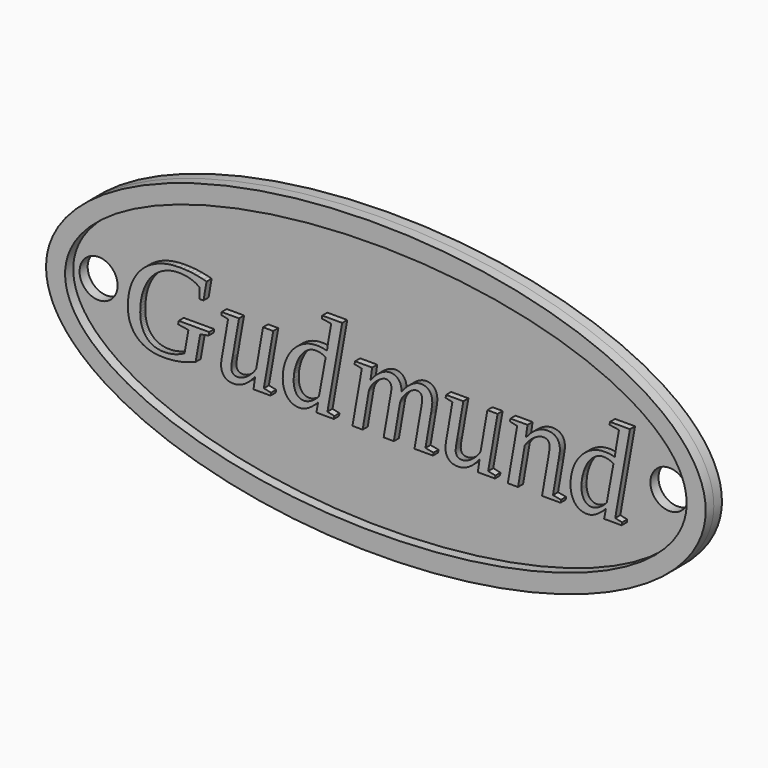
from build123d import *

# Parameters (mm, degrees)
F0_R     = 3
F1_DEPTH = 1.6
F2_DEPTH = 1.6
F3_DEPTH = 1


# Not quite as in the source:
# - a feature names something its author has since deleted; it is built from what else it names


with BuildPart() as f1:
    # F0 (on Front) → F1 (new body)
    with BuildSketch(Plane.XZ):
        with BuildLine():
            add(Edge.make_bspline(
                [(52, 0), (52, 39.8371685741), (-26, 19.918584287), (-104, 0), (-26, -19.918584287), (52, -39.8371685741), (52, 0)],
                knots=[0, 0, 0, 2.0943951024, 2.0943951024, 4.1887902048, 4.1887902048, 6.2831853072, 6.2831853072, 6.2831853072], degree=2, weights=[1, 0.5, 1, 0.5, 1, 0.5, 1]))
        make_face()
        with BuildLine():
            add(Edge.make_bspline(
                [(49, 0), (49, 34.6410161514), (-24.5, 17.3205080757), (-98, 0), (-24.5, -17.3205080757), (49, -34.6410161514), (49, 0)],
                knots=[0, 0, 0, 2.0943951024, 2.0943951024, 4.1887902048, 4.1887902048, 6.2831853072, 6.2831853072, 6.2831853072], degree=2, weights=[1, 0.5, 1, 0.5, 1, 0.5, 1]))
        make_face(mode=Mode.SUBTRACT)
        with BuildLine():
            add(Edge.make_bspline(
                [(49, 0), (49, 34.6410161514), (-24.5, 17.3205080757), (-98, 0), (-24.5, -17.3205080757), (49, -34.6410161514), (49, 0)],
                knots=[0, 0, 0, 2.0943951024, 2.0943951024, 4.1887902048, 4.1887902048, 6.2831853072, 6.2831853072, 6.2831853072], degree=2, weights=[1, 0.5, 1, 0.5, 1, 0.5, 1]))
        make_face()
        Polygon((-28.1758, -1.8651), (-28.9025, -5.9343), (-29.2022, -6.0481), (-29.7981, -6.2613), (-30.0942, -6.3606), (-30.3915, -6.4496), (-30.997, -6.6095), (-31.3052, -6.6803), (-31.6183, -6.7396), (-32.2626, -6.8365), (-32.5938, -6.8741), (-32.9281, -6.9037), (-33.6257, -6.9377), (-33.989, -6.9419), (-34.3187, -6.9363), (-34.6393, -6.9195), (-34.9509, -6.8915), (-35.2533, -6.8523), (-35.5467, -6.8019), (-35.831, -6.7403), (-36.1062, -6.6674), (-36.3724, -6.5834), (-36.6265, -6.4865), (-36.8707, -6.38), (-37.1049, -6.2637), (-37.3291, -6.1377), (-37.5433, -6.0021), (-37.7475, -5.8568), (-37.9418, -5.7018), (-38.126, -5.5371), (-38.2977, -5.363), (-38.459, -5.1798), (-38.6101, -4.9875), (-38.7509, -4.7862), (-38.8814, -4.5758), (-39.0016, -4.3563), (-39.1115, -4.1277), (-39.2111, -3.89), (-39.2974, -3.6438), (-39.3722, -3.3898), (-39.4355, -3.1279), (-39.4872, -2.8582), (-39.5275, -2.5805), (-39.5563, -2.295), (-39.5735, -2.0016), (-39.5793, -1.7004), (-39.5696, -1.2205), (-39.5405, -0.7545), (-39.4921, -0.3025), (-39.4243, 0.1356), (-39.3371, 0.5598), (-39.2305, 0.97), (-39.1046, 1.3664), (-38.9592, 1.7488), (-38.7969, 2.1168), (-38.6201, 2.47), (-38.4288, 2.8083), (-38.2229, 3.1318), (-38.0025, 3.4405), (-37.7675, 3.7343), (-37.518, 4.0133), (-37.254, 4.2775), (-36.9767, 4.5265), (-36.6872, 4.7601), (-36.3857, 4.9782), (-36.072, 5.1809), (-35.7462, 5.3682), (-35.4084, 5.54), (-35.0584, 5.6964), (-34.6962, 5.8373), (-34.322, 5.9622), (-33.9405, 6.0705), (-33.5518, 6.1621), (-33.1558, 6.237), (-32.7525, 6.2953), (-32.3419, 6.3369), (-31.499, 6.3702), (-30.8868, 6.3605), (-30.3001, 6.3315), (-29.7387, 6.283), (-29.2028, 6.2152), (-28.6796, 6.1304), (-27.6623, 5.9173), (-27.1682, 5.7889), (-27.6623, 2.9986), (-28.3115, 2.9986), (-28.2824, 4.6069), (-28.4338, 4.7221), (-28.5924, 4.8303), (-28.7584, 4.9316), (-28.9315, 5.0259), (-29.112, 5.1133), (-29.2997, 5.1937), (-29.4947, 5.2671), (-29.6969, 5.3335), (-29.9062, 5.3948), (-30.122, 5.448), (-30.3446, 5.4929), (-30.5738, 5.5297), (-30.8096, 5.5583), (-31.3013, 5.591), (-31.5571, 5.5951), (-31.8582, 5.5874), (-32.156, 5.5642), (-32.4505, 5.5256), (-32.7416, 5.4716), (-33.0294, 5.4021), (-33.3138, 5.3172), (-33.5949, 5.2168), (-33.8727, 5.101), (-34.1446, 4.9726), (-34.408, 4.8297), (-34.6629, 4.6723), (-34.9094, 4.5003), (-35.1474, 4.3138), (-35.3769, 4.1128), (-35.5979, 3.8972), (-35.8104, 3.6671), (-36.0134, 3.4226), (-36.2058, 3.1639), (-36.3877, 2.891), (-36.5589, 2.6038), (-36.7195, 2.3024), (-36.8695, 1.9867), (-37.0089, 1.6569), (-37.1378, 1.3128), (-37.2536, 0.9575), (-37.3539, 0.5892), (-37.4389, 0.2078), (-37.5084, -0.1865), (-37.5624, -0.5939), (-37.601, -1.0143), (-37.6242, -1.4477), (-37.6319, -1.8941), (-37.6276, -2.1565), (-37.6149, -2.4107), (-37.5937, -2.6567), (-37.5641, -2.8945), (-37.5259, -3.1241), (-37.4793, -3.3456), (-37.4242, -3.5589), (-37.3606, -3.764), (-37.287, -3.9608), (-37.2068, -4.1492), (-37.1199, -4.329), (-37.0263, -4.5004), (-36.9261, -4.6633), (-36.8193, -4.8177), (-36.7057, -4.9636), (-36.5855, -5.1011), (-36.459, -5.2302), (-36.3263, -5.3512), (-36.1877, -5.4639), (-36.043, -5.5685), (-35.8922, -5.665), (-35.7353, -5.7532), (-35.5725, -5.8333), (-35.4035, -5.9052), (-35.2268, -5.9665), (-35.0456, -6.0197), (-34.8599, -6.0646), (-34.6696, -6.1014), (-34.4748, -6.13), (-34.2754, -6.1505), (-34.0715, -6.1627), (-33.863, -6.1668), (-33.6045, -6.162), (-33.352, -6.1474), (-33.1055, -6.1232), (-32.8651, -6.0893), (-32.6314, -6.0433), (-32.1857, -5.9367), (-31.9738, -5.8762), (-31.7703, -5.8071), (-31.5765, -5.7357), (-31.3924, -5.6618), (-31.218, -5.5855), (-31.0552, -5.5086), (-30.9056, -5.4329), (-30.7693, -5.3584), (-30.7062, -5.3216), (-30.6464, -5.2851), (-30.036, -1.8651), (-31.654, -1.6132), (-31.5668, -1.09), (-26.771, -1.09), (-26.8582, -1.6132), align=None, mode=Mode.SUBTRACT)
        Polygon((-23.2726, -4.8675), (-23.2729, -4.8976), (-23.2693, -5.004), (-23.2647, -5.0553), (-23.2584, -5.1053), (-23.2502, -5.154), (-23.2402, -5.2014), (-23.2284, -5.2476), (-23.2148, -5.2924), (-23.1994, -5.336), (-23.1821, -5.3782), (-23.163, -5.4192), (-23.1421, -5.4589), (-23.1194, -5.4974), (-23.0949, -5.5345), (-23.0686, -5.5703), (-23.0404, -5.6049), (-23.0103, -5.6377), (-22.978, -5.6685), (-22.9437, -5.6971), (-22.9072, -5.7236), (-22.8686, -5.7479), (-22.8279, -5.7702), (-22.785, -5.7903), (-22.7401, -5.8083), (-22.693, -5.8242), (-22.6438, -5.838), (-22.5925, -5.8497), (-22.539, -5.8592), (-22.4835, -5.8666), (-22.4258, -5.8719), (-22.366, -5.8751), (-22.3041, -5.8762), (-22.202, -5.8733), (-22.0994, -5.8646), (-21.9961, -5.8503), (-21.8923, -5.8301), (-21.7878, -5.8042), (-21.6828, -5.7726), (-21.5771, -5.7352), (-21.4708, -5.6921), (-21.2601, -5.5934), (-21.0542, -5.4813), (-20.8532, -5.356), (-20.657, -5.2173), (-20.462, -5.0623), (-20.2743, -4.8976), (-20.0939, -4.7232), (-19.9207, -4.5391), (-19.7578, -4.3502), (-19.6082, -4.1613), (-19.472, -3.9723), (-19.349, -3.7834), (-18.2736, 2.3398), (-16.6653, 2.3398), (-18.1477, -6.0893), (-17.0044, -6.3315), (-17.0819, -6.7675), (-19.7753, -6.7675), (-19.5138, -4.8976), (-19.7003, -5.1295), (-20.0878, -5.5607), (-20.2888, -5.7599), (-20.4899, -5.947), (-20.6958, -6.1208), (-20.9065, -6.2813), (-21.1221, -6.4284), (-21.337, -6.5562), (-21.5556, -6.6682), (-21.7779, -6.7645), (-22.0037, -6.845), (-22.2278, -6.9128), (-22.4542, -6.9613), (-22.6831, -6.9903), (-22.9144, -7), (-23.1324, -6.9928), (-23.3407, -6.971), (-23.5394, -6.9346), (-23.635, -6.911), (-23.7283, -6.8838), (-23.8164, -6.8526), (-23.9015, -6.8172), (-23.9835, -6.7775), (-24.0625, -6.7336), (-24.1385, -6.6854), (-24.2115, -6.6331), (-24.2814, -6.5765), (-24.3484, -6.5156), (-24.4097, -6.4507), (-24.4676, -6.3818), (-24.5223, -6.309), (-24.5736, -6.2322), (-24.6216, -6.1515), (-24.6663, -6.0669), (-24.7076, -5.9783), (-24.7456, -5.8858), (-24.7774, -5.7865), (-24.8049, -5.6824), (-24.8282, -5.5734), (-24.8473, -5.4595), (-24.8622, -5.3409), (-24.8728, -5.2173), (-24.8791, -5.089), (-24.8812, -4.9557), (-24.8809, -4.9255), (-24.88, -4.8928), (-24.8785, -4.8576), (-24.8764, -4.8201), (-24.8737, -4.7801), (-24.8703, -4.7377), (-24.8664, -4.6929), (-24.8619, -4.6457), (-24.8473, -4.5464), (-24.8328, -4.4422), (-24.8037, -4.2194), (-24.7843, -4.1025), (-24.7456, -3.8652), (-24.7262, -3.7447), (-24.7026, -3.6205), (-24.659, -3.3832), (-24.639, -3.2699), (-23.7864, 1.6713), (-24.8619, 1.9038), (-24.7843, 2.3398), (-22.0619, 2.3398), (-23.0501, -3.2893), (-23.0695, -3.3971), (-23.1082, -3.6199), (-23.1276, -3.735), (-23.147, -3.8506), (-23.1857, -4.0783), (-23.2051, -4.1903), (-23.219, -4.2993), (-23.2317, -4.4035), (-23.2433, -4.5028), (-23.2535, -4.5973), (-23.2581, -4.6422), (-23.262, -4.6851), (-23.2654, -4.7258), (-23.2681, -4.7644), (-23.2702, -4.8009), (-23.2717, -4.8352), align=None, mode=Mode.SUBTRACT)
        Polygon((3.558, 0.7137), (3.5654, 0.4602), (3.7289, 0.6836), (4.0777, 1.1051), (4.263, 1.3031), (4.4531, 1.4902), (4.6457, 1.664), (4.8407, 1.8245), (5.0381, 1.9716), (5.2373, 2.1085), (5.4377, 2.2283), (5.6394, 2.3313), (5.8422, 2.4173), (5.9461, 2.4559), (6.0493, 2.4893), (6.152, 2.5176), (6.254, 2.5408), (6.3554, 2.5588), (6.4562, 2.5717), (6.5565, 2.5794), (6.6561, 2.582), (6.7564, 2.5799), (6.8541, 2.5738), (6.949, 2.5636), (7.0412, 2.5493), (7.1307, 2.5309), (7.2174, 2.5084), (7.3014, 2.4818), (7.3827, 2.4512), (7.4613, 2.4164), (7.5371, 2.3776), (7.6102, 2.3347), (7.6806, 2.2877), (7.7483, 2.2366), (7.8133, 2.1814), (7.8755, 2.1222), (7.935, 2.0588), (7.9925, 1.9928), (8.0462, 1.9232), (8.0963, 1.8499), (8.1427, 1.773), (8.1853, 1.6924), (8.2243, 1.6083), (8.2595, 1.5205), (8.291, 1.429), (8.3188, 1.334), (8.3429, 1.2353), (8.3633, 1.1329), (8.38, 1.027), (8.393, 0.9174), (8.4023, 0.8041), (8.4079, 0.6873), (8.4097, 0.5668), (8.4094, 0.5295), (8.4085, 0.4905), (8.407, 0.4496), (8.4049, 0.4069), (8.3988, 0.3161), (8.3903, 0.218), (8.3794, 0.1144), (8.3504, -0.1036), (8.3322, -0.218), (8.3171, -0.3349), (8.2831, -0.5723), (8.2644, -0.6928), (8.245, -0.812), (8.2062, -1.0397), (8.1869, -1.1481), (7.3343, -6.0893), (8.6035, -6.3315), (8.5163, -6.7675), (5.6, -6.7675), (6.5979, -1.1287), (6.6173, -1.0252), (6.6561, -0.8072), (6.6754, -0.6928), (6.6942, -0.5729), (6.7281, -0.3403), (6.7433, -0.2277), (6.7614, -0.1187), (6.7772, -0.0146), (6.7905, 0.0847), (6.8014, 0.1792), (6.8059, 0.2242), (6.8099, 0.267), (6.8132, 0.3077), (6.8159, 0.3463), (6.8181, 0.3828), (6.8196, 0.4172), (6.8205, 0.4494), (6.8208, 0.4796), (6.8176, 0.5858), (6.8081, 0.6867), (6.7922, 0.782), (6.7818, 0.8277), (6.7699, 0.8719), (6.7564, 0.9149), (6.7413, 0.9564), (6.7246, 0.9966), (6.7063, 1.0354), (6.6865, 1.0729), (6.665, 1.109), (6.642, 1.1438), (6.6173, 1.1771), (6.591, 1.21), (6.5628, 1.2407), (6.5328, 1.2693), (6.5011, 1.2958), (6.4674, 1.3202), (6.432, 1.3424), (6.3948, 1.3626), (6.3557, 1.3806), (6.3149, 1.3965), (6.2722, 1.4103), (6.2277, 1.4219), (6.1813, 1.4315), (6.1332, 1.4389), (6.0832, 1.4442), (6.0315, 1.4474), (5.9779, 1.4484), (5.9214, 1.4466), (5.8634, 1.4412), (5.8039, 1.4321), (5.7429, 1.4194), (5.6804, 1.403), (5.6164, 1.383), (5.5508, 1.3594), (5.4838, 1.3322), (5.3475, 1.2686), (5.2101, 1.1941), (5.0714, 1.1087), (4.9315, 1.0124), (4.7916, 0.9113), (4.653, 0.8017), (4.5155, 0.6836), (4.3793, 0.5571), (4.2509, 0.4245), (4.0087, 0.1483), (3.8948, 0.0048), (3.7876, -0.1417), (3.6889, -0.2907), (3.5987, -0.4421), (3.517, -0.5959), (3.4461, -0.7491), (3.3886, -0.8986), (3.3648, -0.9721), (3.3444, -1.0446), (3.3273, -1.1162), (3.3135, -1.1869), (2.3543, -6.7675), (0.746, -6.7675), (1.7343, -1.1287), (1.7536, -1.0252), (1.7924, -0.8072), (1.8118, -0.6928), (1.8312, -0.5729), (1.8699, -0.3403), (1.8893, -0.2277), (1.9075, -0.1187), (1.9232, -0.0146), (1.9365, 0.0847), (1.9474, 0.1792), (1.9542, 0.2242), (1.9601, 0.267), (1.9651, 0.3077), (1.9692, 0.3463), (1.9724, 0.3828), (1.9747, 0.4172), (1.976, 0.4494), (1.9765, 0.4796), (1.9732, 0.5858), (1.9632, 0.6867), (1.9557, 0.735), (1.9465, 0.782), (1.9357, 0.8277), (1.9232, 0.8719), (1.909, 0.9149), (1.8932, 0.9564), (1.8757, 0.9966), (1.8566, 1.0354), (1.8358, 1.0729), (1.8133, 1.109), (1.7891, 1.1438), (1.7633, 1.1771), (1.7357, 1.21), (1.7063, 1.2407), (1.6749, 1.2693), (1.6416, 1.2958), (1.6065, 1.3202), (1.5694, 1.3424), (1.5305, 1.3626), (1.4896, 1.3806), (1.4469, 1.3965), (1.4023, 1.4103), (1.3558, 1.4219), (1.3074, 1.4315), (1.2571, 1.4389), (1.2049, 1.4442), (1.1508, 1.4474), (1.0948, 1.4484), (1.0384, 1.4466), (0.9804, 1.4412), (0.9209, 1.4321), (0.8599, 1.4194), (0.7974, 1.403), (0.7333, 1.383), (0.6678, 1.3594), (0.6007, 1.3322), (0.4639, 1.2686), (0.3246, 1.1941), (0.1829, 1.1087), (0.0388, 1.0124), (-0.1017, 0.9113), (-0.2422, 0.8017), (-0.3827, 0.6836), (-0.5232, 0.5571), (-0.6564, 0.4245), (-0.9083, 0.1483), (-1.027, 0.0048), (-1.1342, -0.1417), (-1.2329, -0.2907), (-1.3231, -0.4421), (-1.4048, -0.5959), (-1.4757, -0.7491), (-1.5332, -0.8986), (-1.557, -0.9721), (-1.5774, -1.0446), (-1.5945, -1.1162), (-1.6083, -1.1869), (-2.5675, -6.7675), (-4.1758, -6.7675), (-2.6934, 1.6616), (-3.8367, 1.9038), (-3.7592, 2.3398), (-1.0657, 2.3398), (-1.337, 0.4602), (-1.1735, 0.6836), (-0.8247, 1.1051), (-0.6394, 1.3031), (-0.4487, 1.4902), (-0.2543, 1.664), (-0.0563, 1.8245), (0.1453, 1.9716), (0.3488, 2.1085), (0.5523, 2.2283), (0.7557, 2.3313), (0.9592, 2.4173), (1.063, 2.4559), (1.1663, 2.4893), (1.2689, 2.5176), (1.371, 2.5408), (1.4724, 2.5588), (1.5732, 2.5717), (1.6734, 2.5794), (1.773, 2.582), (1.8781, 2.5799), (1.9801, 2.5735), (2.0791, 2.5629), (2.1751, 2.5481), (2.2681, 2.529), (2.358, 2.5057), (2.4449, 2.4781), (2.5287, 2.4463), (2.6096, 2.4103), (2.6874, 2.37), (2.7622, 2.3255), (2.8339, 2.2768), (2.9027, 2.2238), (2.9684, 2.1666), (3.031, 2.1051), (3.0907, 2.0394), (3.1482, 1.9708), (3.2019, 1.8982), (3.252, 1.8215), (3.2984, 1.7409), (3.341, 1.6562), (3.38, 1.5676), (3.4152, 1.4749), (3.4467, 1.3782), (3.4745, 1.2775), (3.4987, 1.1727), (3.5191, 1.064), (3.5357, 0.9513), (3.5487, 0.8345), align=None, mode=Mode.SUBTRACT)
        Polygon((12.1018, -4.8675), (12.1015, -4.8976), (12.1052, -5.004), (12.1097, -5.0553), (12.1161, -5.1053), (12.1242, -5.154), (12.1342, -5.2014), (12.146, -5.2476), (12.1597, -5.2924), (12.1751, -5.336), (12.1924, -5.3782), (12.2114, -5.4192), (12.2323, -5.4589), (12.255, -5.4974), (12.2796, -5.5345), (12.3059, -5.5703), (12.3341, -5.6049), (12.3642, -5.6377), (12.3964, -5.6685), (12.4308, -5.6971), (12.4673, -5.7236), (12.5059, -5.7479), (12.5466, -5.7702), (12.5894, -5.7903), (12.6344, -5.8083), (12.6815, -5.8242), (12.7307, -5.838), (12.782, -5.8497), (12.8354, -5.8592), (12.891, -5.8666), (12.9487, -5.8719), (13.0085, -5.8751), (13.0704, -5.8762), (13.1724, -5.8733), (13.2751, -5.8646), (13.3783, -5.8503), (13.4822, -5.8301), (13.5866, -5.8042), (13.6917, -5.7726), (13.7973, -5.7352), (13.9036, -5.6921), (14.1143, -5.5934), (14.3202, -5.4813), (14.5213, -5.356), (14.7175, -5.2173), (14.9124, -5.0623), (15.1002, -4.8976), (15.2806, -4.7232), (15.4538, -4.5391), (15.6167, -4.3502), (15.7662, -4.1613), (15.9025, -3.9723), (16.0254, -3.7834), (17.1008, 2.3398), (18.7092, 2.3398), (17.2268, -6.0893), (18.3701, -6.3315), (18.2925, -6.7675), (15.5991, -6.7675), (15.8607, -4.8976), (15.6742, -5.1295), (15.2867, -5.5607), (15.0856, -5.7599), (14.8846, -5.947), (14.6787, -6.1208), (14.468, -6.2813), (14.2524, -6.4284), (14.0374, -6.5562), (13.8188, -6.6682), (13.5966, -6.7645), (13.3707, -6.845), (13.1467, -6.9128), (12.9202, -6.9613), (12.6913, -6.9903), (12.46, -7), (12.242, -6.9928), (12.0337, -6.971), (11.8351, -6.9346), (11.7394, -6.911), (11.6462, -6.8838), (11.5581, -6.8526), (11.473, -6.8172), (11.3909, -6.7775), (11.3119, -6.7336), (11.2359, -6.6854), (11.163, -6.6331), (11.093, -6.5765), (11.0261, -6.5156), (10.9648, -6.4507), (10.9068, -6.3818), (10.8522, -6.309), (10.8008, -6.2322), (10.7529, -6.1515), (10.7082, -6.0669), (10.6669, -5.9783), (10.6289, -5.8858), (10.5971, -5.7865), (10.5695, -5.6824), (10.5462, -5.5734), (10.5271, -5.4595), (10.5123, -5.3409), (10.5017, -5.2173), (10.4954, -5.089), (10.4932, -4.9557), (10.4935, -4.9255), (10.4944, -4.8928), (10.496, -4.8576), (10.4981, -4.8201), (10.5008, -4.7801), (10.5041, -4.7377), (10.5081, -4.6929), (10.5126, -4.6457), (10.5271, -4.5464), (10.5417, -4.4422), (10.5707, -4.2194), (10.5901, -4.1025), (10.6289, -3.8652), (10.6483, -3.7447), (10.6719, -3.6205), (10.7155, -3.3832), (10.7354, -3.2699), (11.588, 1.6713), (10.5126, 1.9038), (10.5901, 2.3398), (13.3126, 2.3398), (12.3244, -3.2893), (12.305, -3.3971), (12.2662, -3.6199), (12.2469, -3.735), (12.2275, -3.8506), (12.1887, -4.0783), (12.1694, -4.1903), (12.1554, -4.2993), (12.1427, -4.4035), (12.1312, -4.5028), (12.1209, -4.5973), (12.1164, -4.6422), (12.1124, -4.6851), (12.1091, -4.7258), (12.1064, -4.7644), (12.1043, -4.8009), (12.1028, -4.8352), align=None, mode=Mode.SUBTRACT)
        Polygon((26.9252, 0.4494), (26.9256, 0.4796), (26.9219, 0.586), (26.9174, 0.6373), (26.911, 0.6873), (26.9028, 0.736), (26.8929, 0.7834), (26.881, 0.8295), (26.8674, 0.8744), (26.852, 0.9179), (26.8347, 0.9602), (26.8156, 1.0012), (26.7948, 1.0409), (26.772, 1.0793), (26.7475, 1.1164), (26.7212, 1.1523), (26.693, 1.1868), (26.6629, 1.2197), (26.6307, 1.2504), (26.5963, 1.279), (26.5598, 1.3055), (26.5212, 1.3299), (26.4805, 1.3521), (26.4376, 1.3723), (26.3927, 1.3903), (26.3456, 1.4062), (26.2964, 1.42), (26.2451, 1.4316), (26.1916, 1.4412), (26.1361, 1.4486), (26.0784, 1.4539), (26.0186, 1.457), (25.9567, 1.4581), (25.8547, 1.4551), (25.752, 1.446), (25.6488, 1.4309), (25.5449, 1.4097), (25.4405, 1.3824), (25.3354, 1.3491), (25.2297, 1.3097), (25.1235, 1.2643), (24.9121, 1.165), (24.7044, 1.0512), (24.5004, 0.9228), (24.2999, 0.7799), (24.105, 0.6243), (23.9172, 0.4578), (23.7368, 0.2803), (23.5636, 0.092), (23.4007, -0.0969), (23.2512, -0.2858), (23.1149, -0.4748), (22.992, -0.6637), (21.9262, -6.7675), (20.3179, -6.7675), (21.8003, 1.6713), (20.657, 1.9135), (20.7345, 2.3495), (23.428, 2.3495), (23.1664, 0.4892), (23.3523, 0.7212), (23.735, 1.1523), (23.9318, 1.3515), (24.1365, 1.538), (24.3435, 1.71), (24.5531, 1.8674), (24.765, 2.0104), (24.9836, 2.1381), (25.2034, 2.2501), (25.4244, 2.3464), (25.6467, 2.427), (25.8749, 2.4948), (26.1044, 2.5432), (26.3352, 2.5723), (26.5671, 2.582), (26.7845, 2.5747), (26.8891, 2.5656), (26.9909, 2.5529), (27.0901, 2.5366), (27.1865, 2.5166), (27.2802, 2.493), (27.3712, 2.4657), (27.4615, 2.4345), (27.548, 2.3991), (27.631, 2.3594), (27.7103, 2.3155), (27.786, 2.2674), (27.8581, 2.215), (27.9265, 2.1584), (27.9913, 2.0976), (28.0547, 2.0325), (28.1142, 1.9631), (28.1698, 1.8895), (28.2214, 1.8117), (28.2691, 1.7297), (28.3128, 1.6434), (28.3526, 1.5529), (28.3885, 1.4581), (28.4226, 1.3589), (28.4521, 1.2553), (28.4771, 1.147), (28.4975, 1.0342), (28.5134, 0.9169), (28.5248, 0.795), (28.5316, 0.6686), (28.5339, 0.5377), (28.5337, 0.5228), (28.5334, 0.5073), (28.532, 0.4741), (28.5298, 0.4382), (28.5266, 0.3996), (28.5225, 0.3583), (28.5175, 0.3142), (28.5116, 0.2675), (28.5048, 0.218), (28.4939, 0.1187), (28.4806, 0.0145), (28.4648, -0.0945), (28.4467, -0.2083), (28.4273, -0.3258), (28.3885, -0.568), (28.3691, -0.6928), (28.3498, -0.812), (28.311, -1.0397), (28.2916, -1.1481), (27.439, -6.099), (28.7083, -6.3315), (28.6307, -6.7675), (25.7145, -6.7675), (26.7027, -1.1287), (26.7221, -1.021), (26.7608, -0.7981), (26.7802, -0.6831), (26.799, -0.5674), (26.8329, -0.3397), (26.848, -0.2277), (26.8662, -0.1187), (26.882, -0.0146), (26.8953, 0.0847), (26.9062, 0.1792), (26.9107, 0.2242), (26.9147, 0.267), (26.918, 0.3077), (26.9207, 0.3463), (26.9228, 0.3828), (26.9243, 0.4172), align=None, mode=Mode.SUBTRACT)
        with Locations((-45, 0)):
            Circle(F0_R, mode=Mode.SUBTRACT)
        Polygon((-8.3466, 2.3997), (-8.1776, 2.3495), (-8.1763, 2.3644), (-8.1749, 2.38), (-8.1733, 2.3965), (-8.1716, 2.4136), (-8.1676, 2.4503), (-8.1631, 2.4899), (-8.158, 2.5326), (-8.1522, 2.5783), (-8.1458, 2.6271), (-8.1389, 2.6789), (-8.1237, 2.7909), (-8.0898, 3.0186), (-8.0711, 3.1342), (-8.0523, 3.2541), (-8.0184, 3.4867), (-8.0032, 3.5993), (-7.9937, 3.6538), (-7.9845, 3.7059), (-7.9755, 3.7555), (-7.9669, 3.8027), (-7.9586, 3.8476), (-7.9506, 3.8899), (-7.9428, 3.9299), (-7.9354, 3.9674), (-7.5188, 6.3315), (-9.0108, 6.564), (-8.9333, 7), (-5.7942, 7), (-8.1195, -6.0893), (-7.0247, -6.3315), (-7.1022, -6.7675), (-9.8634, -6.7675), (-9.5825, -5.2561), (-9.7849, -5.4627), (-9.9852, -5.6563), (-10.1833, -5.8369), (-10.3794, -6.0045), (-10.5733, -6.1591), (-10.7651, -6.3006), (-10.9548, -6.4292), (-11.1423, -6.5447), (-11.3279, -6.6446), (-11.5117, -6.7312), (-11.6937, -6.8044), (-11.8738, -6.8644), (-12.0522, -6.911), (-12.2287, -6.9443), (-12.4034, -6.9643), (-12.5762, -6.971), (-12.7199, -6.9675), (-12.8602, -6.957), (-12.9972, -6.9396), (-13.1309, -6.9153), (-13.2613, -6.8839), (-13.3883, -6.8456), (-13.512, -6.8004), (-13.6323, -6.7481), (-13.7489, -6.6894), (-13.8612, -6.6246), (-13.9693, -6.5537), (-14.0731, -6.4768), (-14.1727, -6.3939), (-14.2681, -6.3049), (-14.3592, -6.2098), (-14.4461, -6.1087), (-14.5286, -5.9992), (-14.6066, -5.884), (-14.68, -5.7631), (-14.7489, -5.6364), (-14.8132, -5.5039), (-14.873, -5.3657), (-14.9283, -5.2217), (-14.979, -5.072), (-15.0222, -4.917), (-15.0596, -4.7571), (-15.0912, -4.5924), (-15.1372, -4.2485), (-15.1602, -3.8851), (-15.1631, -3.6962), (-15.1516, -3.2826), (-15.1171, -2.8751), (-15.0596, -2.4736), (-14.979, -2.0782), (-14.8773, -1.6871), (-14.7562, -1.308), (-14.6157, -0.941), (-14.4558, -0.5862), (-14.2778, -0.2453), (-14.0828, 0.0799), (-13.8709, 0.3893), (-13.642, 0.683), (-13.3925, 0.9634), (-13.1285, 1.2232), (-12.8499, 1.4623), (-12.5569, 1.6809), (-12.2505, 1.882), (-11.932, 2.0588), (-11.6013, 2.2114), (-11.2586, 2.3398), (-10.9007, 2.4415), (-10.5344, 2.5142), (-10.1596, 2.5578), (-9.7762, 2.5723), (-9.5401, 2.5687), (-9.316, 2.5578), (-9.1041, 2.5396), (-8.9043, 2.5142), (-8.7099, 2.4821), (-8.524, 2.4439), align=None, mode=Mode.SUBTRACT)
        Polygon((37.027, 2.3997), (37.1959, 2.3495), (37.1972, 2.3644), (37.1987, 2.38), (37.2002, 2.3965), (37.202, 2.4136), (37.2059, 2.4503), (37.2105, 2.4899), (37.2156, 2.5326), (37.2214, 2.5783), (37.2277, 2.6271), (37.2347, 2.6789), (37.2498, 2.7909), (37.2837, 3.0186), (37.3025, 3.1342), (37.3213, 3.2541), (37.3552, 3.4867), (37.3703, 3.5993), (37.3799, 3.6538), (37.3891, 3.7059), (37.398, 3.7555), (37.4067, 3.8027), (37.415, 3.8476), (37.423, 3.8899), (37.4307, 3.9299), (37.4381, 3.9674), (37.8548, 6.3315), (36.3627, 6.564), (36.4402, 7), (39.5793, 7), (37.2541, -6.0893), (38.3489, -6.3315), (38.2714, -6.7675), (35.5101, -6.7675), (35.7911, -5.2561), (35.5887, -5.4627), (35.3884, -5.6563), (35.1902, -5.8369), (34.9942, -6.0045), (34.8003, -6.1591), (34.6085, -6.3006), (34.4188, -6.4292), (34.2312, -6.5447), (34.0456, -6.6446), (33.8618, -6.7312), (33.6799, -6.8044), (33.4997, -6.8644), (33.3214, -6.911), (33.1449, -6.9443), (32.9702, -6.9643), (32.7973, -6.971), (32.6537, -6.9675), (32.5133, -6.957), (32.3763, -6.9396), (32.2426, -6.9153), (32.1123, -6.8839), (31.9853, -6.8456), (31.8616, -6.8004), (31.7413, -6.7481), (31.6247, -6.6894), (31.5124, -6.6246), (31.4043, -6.5537), (31.3004, -6.4768), (31.2008, -6.3939), (31.1054, -6.3049), (31.0143, -6.2098), (30.9274, -6.1087), (30.8449, -5.9992), (30.767, -5.884), (30.6935, -5.7631), (30.6247, -5.6364), (30.5603, -5.5039), (30.5005, -5.3657), (30.4453, -5.2217), (30.3945, -5.072), (30.3514, -4.917), (30.314, -4.7571), (30.2824, -4.5924), (30.2364, -4.2485), (30.2133, -3.8851), (30.2105, -3.6962), (30.222, -3.2826), (30.2565, -2.8751), (30.314, -2.4736), (30.3945, -2.0782), (30.4963, -1.6871), (30.6174, -1.308), (30.7579, -0.941), (30.9177, -0.5862), (31.0958, -0.2453), (31.2907, 0.0799), (31.5027, 0.3893), (31.7316, 0.683), (31.9811, 0.9634), (32.2451, 1.2232), (32.5236, 1.4623), (32.8167, 1.6809), (33.1231, 1.882), (33.4416, 2.0588), (33.7722, 2.2114), (34.115, 2.3398), (34.4728, 2.4415), (34.8392, 2.5142), (35.214, 2.5578), (35.5973, 2.5723), (35.8335, 2.5687), (36.0575, 2.5578), (36.2695, 2.5396), (36.4693, 2.5142), (36.6637, 2.4821), (36.8496, 2.4439), align=None, mode=Mode.SUBTRACT)
        with Locations((45, 0)):
            Circle(F0_R, mode=Mode.SUBTRACT)
        Polygon((-8.1763, 2.3644), (-8.1776, 2.3495), (-8.3466, 2.3997), (-8.524, 2.4439), (-8.7099, 2.4821), (-8.9043, 2.5142), (-9.1041, 2.5396), (-9.316, 2.5578), (-9.5401, 2.5687), (-9.7762, 2.5723), (-10.1596, 2.5578), (-10.5344, 2.5142), (-10.9007, 2.4415), (-11.2586, 2.3398), (-11.6013, 2.2114), (-11.932, 2.0588), (-12.2505, 1.882), (-12.5569, 1.6809), (-12.8499, 1.4623), (-13.1285, 1.2232), (-13.3925, 0.9634), (-13.642, 0.683), (-13.8709, 0.3893), (-14.0828, 0.0799), (-14.2778, -0.2453), (-14.4558, -0.5862), (-14.6157, -0.941), (-14.7562, -1.308), (-14.8773, -1.6871), (-14.979, -2.0782), (-15.0596, -2.4736), (-15.1171, -2.8751), (-15.1516, -3.2826), (-15.1631, -3.6962), (-15.1602, -3.8851), (-15.1372, -4.2485), (-15.0912, -4.5924), (-15.0596, -4.7571), (-15.0222, -4.917), (-14.979, -5.072), (-14.9283, -5.2217), (-14.873, -5.3657), (-14.8132, -5.5039), (-14.7489, -5.6364), (-14.68, -5.7631), (-14.6066, -5.884), (-14.5286, -5.9992), (-14.4461, -6.1087), (-14.3592, -6.2098), (-14.2681, -6.3049), (-14.1727, -6.3939), (-14.0731, -6.4768), (-13.9693, -6.5537), (-13.8612, -6.6246), (-13.7489, -6.6894), (-13.6323, -6.7481), (-13.512, -6.8004), (-13.3883, -6.8456), (-13.2613, -6.8839), (-13.1309, -6.9153), (-12.9972, -6.9396), (-12.8602, -6.957), (-12.7199, -6.9675), (-12.5762, -6.971), (-12.4034, -6.9643), (-12.2287, -6.9443), (-12.0522, -6.911), (-11.8738, -6.8644), (-11.6937, -6.8044), (-11.5117, -6.7312), (-11.3279, -6.6446), (-11.1423, -6.5447), (-10.9548, -6.4292), (-10.7651, -6.3006), (-10.5733, -6.1591), (-10.3794, -6.0045), (-10.1833, -5.8369), (-9.9852, -5.6563), (-9.7849, -5.4627), (-9.5825, -5.2561), (-9.8634, -6.7675), (-7.1022, -6.7675), (-7.0247, -6.3315), (-8.1195, -6.0893), (-5.7942, 7), (-8.9333, 7), (-9.0108, 6.564), (-7.5188, 6.3315), (-7.9354, 3.9674), (-7.9428, 3.9299), (-7.9506, 3.8899), (-7.9586, 3.8476), (-7.9669, 3.8027), (-7.9755, 3.7555), (-7.9845, 3.7059), (-7.9937, 3.6538), (-8.0032, 3.5993), (-8.0184, 3.4867), (-8.0523, 3.2541), (-8.0711, 3.1342), (-8.0898, 3.0186), (-8.1237, 2.7909), (-8.1389, 2.6789), (-8.1458, 2.6271), (-8.1522, 2.5783), (-8.158, 2.5326), (-8.1631, 2.4899), (-8.1676, 2.4503), (-8.1716, 2.4136), (-8.1733, 2.3965), (-8.1749, 2.38), align=None)
        Polygon((-8.5712, 1.4472), (-8.4005, 1.3418), (-9.4565, -4.4132), (-9.605, -4.5686), (-9.9066, -4.8532), (-10.0596, -4.9824), (-10.2142, -5.1027), (-10.3703, -5.2143), (-10.5279, -5.3171), (-10.687, -5.4111), (-10.843, -5.4928), (-10.9964, -5.5637), (-11.147, -5.6236), (-11.2949, -5.6727), (-11.4401, -5.7108), (-11.5826, -5.7381), (-11.7223, -5.7544), (-11.8593, -5.7599), (-11.9342, -5.7579), (-12.0089, -5.752), (-12.0832, -5.7422), (-12.1572, -5.7284), (-12.2309, -5.7107), (-12.3044, -5.689), (-12.3775, -5.6635), (-12.4503, -5.6339), (-12.5196, -5.6002), (-12.5871, -5.5619), (-12.6528, -5.519), (-12.7167, -5.4717), (-12.7788, -5.4197), (-12.839, -5.3633), (-12.8975, -5.3023), (-12.9541, -5.2367), (-13.0062, -5.1642), (-13.0558, -5.0871), (-13.1031, -5.0055), (-13.1479, -4.9194), (-13.1903, -4.8287), (-13.2302, -4.7335), (-13.2678, -4.6337), (-13.3029, -4.5294), (-13.3347, -4.4177), (-13.3622, -4.3005), (-13.3855, -4.1779), (-13.4046, -4.0499), (-13.4195, -3.9163), (-13.4301, -3.7774), (-13.4364, -3.6329), (-13.4385, -3.4831), (-13.4319, -3.1724), (-13.3786, -2.5475), (-13.332, -2.2332), (-13.2678, -1.9208), (-13.1031, -1.3104), (-13.0025, -1.0125), (-12.8905, -0.7218), (-12.7676, -0.4409), (-12.6338, -0.1696), (-12.489, 0.092), (-12.3292, 0.3403), (-12.1596, 0.5716), (-11.9804, 0.786), (-11.7915, 0.9834), (-11.6935, 1.0777), (-11.4913, 1.2509), (-11.2806, 1.4035), (-11.0613, 1.5355), (-10.9486, 1.5937), (-10.8337, 1.646), (-10.7166, 1.6912), (-10.5975, 1.7295), (-10.4762, 1.7609), (-10.3529, 1.7852), (-10.2274, 1.8027), (-10.0998, 1.8131), (-9.97, 1.8166), (-9.8441, 1.8146), (-9.723, 1.8087), (-9.6067, 1.7989), (-9.4953, 1.7851), (-9.3887, 1.7674), (-9.287, 1.7457), (-9.1901, 1.7202), (-9.098, 1.6906), (-8.92, 1.6216), (-8.7444, 1.5405), align=None, mode=Mode.SUBTRACT)
        Polygon((37.1972, 2.3644), (37.1959, 2.3495), (37.027, 2.3997), (36.8496, 2.4439), (36.6637, 2.4821), (36.4693, 2.5142), (36.2695, 2.5396), (36.0575, 2.5578), (35.8335, 2.5687), (35.5973, 2.5723), (35.214, 2.5578), (34.8392, 2.5142), (34.4728, 2.4415), (34.115, 2.3398), (33.7722, 2.2114), (33.4416, 2.0588), (33.1231, 1.882), (32.8167, 1.6809), (32.5236, 1.4623), (32.2451, 1.2232), (31.9811, 0.9634), (31.7316, 0.683), (31.5027, 0.3893), (31.2907, 0.0799), (31.0958, -0.2453), (30.9177, -0.5862), (30.7579, -0.941), (30.6174, -1.308), (30.4963, -1.6871), (30.3945, -2.0782), (30.314, -2.4736), (30.2565, -2.8751), (30.222, -3.2826), (30.2105, -3.6962), (30.2133, -3.8851), (30.2364, -4.2485), (30.2824, -4.5924), (30.314, -4.7571), (30.3514, -4.917), (30.3945, -5.072), (30.4453, -5.2217), (30.5005, -5.3657), (30.5603, -5.5039), (30.6247, -5.6364), (30.6935, -5.7631), (30.767, -5.884), (30.8449, -5.9992), (30.9274, -6.1087), (31.0143, -6.2098), (31.1054, -6.3049), (31.2008, -6.3939), (31.3004, -6.4768), (31.4043, -6.5537), (31.5124, -6.6246), (31.6247, -6.6894), (31.7413, -6.7481), (31.8616, -6.8004), (31.9853, -6.8456), (32.1123, -6.8839), (32.2426, -6.9153), (32.3763, -6.9396), (32.5133, -6.957), (32.6537, -6.9675), (32.7973, -6.971), (32.9702, -6.9643), (33.1449, -6.9443), (33.3214, -6.911), (33.4997, -6.8644), (33.6799, -6.8044), (33.8618, -6.7312), (34.0456, -6.6446), (34.2312, -6.5447), (34.4188, -6.4292), (34.6085, -6.3006), (34.8003, -6.1591), (34.9942, -6.0045), (35.1902, -5.8369), (35.3884, -5.6563), (35.5887, -5.4627), (35.7911, -5.2561), (35.5101, -6.7675), (38.2714, -6.7675), (38.3489, -6.3315), (37.2541, -6.0893), (39.5793, 7), (36.4402, 7), (36.3627, 6.564), (37.8548, 6.3315), (37.4381, 3.9674), (37.4307, 3.9299), (37.423, 3.8899), (37.415, 3.8476), (37.4067, 3.8027), (37.398, 3.7555), (37.3891, 3.7059), (37.3799, 3.6538), (37.3703, 3.5993), (37.3552, 3.4867), (37.3213, 3.2541), (37.3025, 3.1342), (37.2837, 3.0186), (37.2498, 2.7909), (37.2347, 2.6789), (37.2277, 2.6271), (37.2214, 2.5783), (37.2156, 2.5326), (37.2105, 2.4899), (37.2059, 2.4503), (37.202, 2.4136), (37.2002, 2.3965), (37.1987, 2.38), align=None)
        Polygon((36.8023, 1.4472), (36.9731, 1.3418), (35.917, -4.4132), (35.7685, -4.5686), (35.467, -4.8532), (35.3139, -4.9824), (35.1594, -5.1027), (35.0033, -5.2143), (34.8457, -5.3171), (34.6866, -5.4111), (34.5305, -5.4928), (34.3772, -5.5637), (34.2265, -5.6236), (34.0786, -5.6727), (33.9335, -5.7108), (33.791, -5.7381), (33.6513, -5.7544), (33.5143, -5.7599), (33.4393, -5.7579), (33.3647, -5.752), (33.2904, -5.7422), (33.2163, -5.7284), (33.1426, -5.7107), (33.0692, -5.689), (32.9961, -5.6635), (32.9233, -5.6339), (32.8539, -5.6002), (32.7864, -5.5619), (32.7207, -5.519), (32.6568, -5.4717), (32.5948, -5.4197), (32.5345, -5.3633), (32.4761, -5.3023), (32.4195, -5.2367), (32.3674, -5.1642), (32.3177, -5.0871), (32.2705, -5.0055), (32.2257, -4.9194), (32.1833, -4.8287), (32.1433, -4.7335), (32.1058, -4.6337), (32.0707, -4.5294), (32.0389, -4.4177), (32.0113, -4.3005), (31.988, -4.1779), (31.9689, -4.0499), (31.9541, -3.9163), (31.9435, -3.7774), (31.9372, -3.6329), (31.935, -3.4831), (31.9417, -3.1724), (31.995, -2.5475), (32.0416, -2.2332), (32.1058, -1.9208), (32.2705, -1.3104), (32.371, -1.0125), (32.483, -0.7218), (32.606, -0.4409), (32.7398, -0.1696), (32.8845, 0.092), (33.0444, 0.3403), (33.2139, 0.5716), (33.3932, 0.786), (33.5821, 0.9834), (33.68, 1.0777), (33.8823, 1.2509), (34.093, 1.4035), (34.3122, 1.5355), (34.425, 1.5937), (34.5399, 1.646), (34.6569, 1.6912), (34.7761, 1.7295), (34.8973, 1.7609), (35.0207, 1.7852), (35.1462, 1.8027), (35.2738, 1.8131), (35.4035, 1.8166), (35.5295, 1.8146), (35.6506, 1.8087), (35.7669, 1.7989), (35.8783, 1.7851), (35.9849, 1.7674), (36.0866, 1.7457), (36.1835, 1.7202), (36.2755, 1.6906), (36.4535, 1.6216), (36.6292, 1.5405), align=None, mode=Mode.SUBTRACT)
        Polygon((3.7289, 0.6836), (3.5654, 0.4602), (3.558, 0.7137), (3.5487, 0.8345), (3.5357, 0.9513), (3.5191, 1.064), (3.4987, 1.1727), (3.4745, 1.2775), (3.4467, 1.3782), (3.4152, 1.4749), (3.38, 1.5676), (3.341, 1.6562), (3.2984, 1.7409), (3.252, 1.8215), (3.2019, 1.8982), (3.1482, 1.9708), (3.0907, 2.0394), (3.031, 2.1051), (2.9684, 2.1666), (2.9027, 2.2238), (2.8339, 2.2768), (2.7622, 2.3255), (2.6874, 2.37), (2.6096, 2.4103), (2.5287, 2.4463), (2.4449, 2.4781), (2.358, 2.5057), (2.2681, 2.529), (2.1751, 2.5481), (2.0791, 2.5629), (1.9801, 2.5735), (1.8781, 2.5799), (1.773, 2.582), (1.6734, 2.5794), (1.5732, 2.5717), (1.4724, 2.5588), (1.371, 2.5408), (1.2689, 2.5176), (1.1663, 2.4893), (1.063, 2.4559), (0.9592, 2.4173), (0.7557, 2.3313), (0.5523, 2.2283), (0.3488, 2.1085), (0.1453, 1.9716), (-0.0563, 1.8245), (-0.2543, 1.664), (-0.4487, 1.4902), (-0.6394, 1.3031), (-0.8247, 1.1051), (-1.1735, 0.6836), (-1.337, 0.4602), (-1.0657, 2.3398), (-3.7592, 2.3398), (-3.8367, 1.9038), (-2.6934, 1.6616), (-4.1758, -6.7675), (-2.5675, -6.7675), (-1.6083, -1.1869), (-1.5945, -1.1162), (-1.5774, -1.0446), (-1.557, -0.9721), (-1.5332, -0.8986), (-1.4757, -0.7491), (-1.4048, -0.5959), (-1.3231, -0.4421), (-1.2329, -0.2907), (-1.1342, -0.1417), (-1.027, 0.0048), (-0.9083, 0.1483), (-0.6564, 0.4245), (-0.5232, 0.5571), (-0.3827, 0.6836), (-0.2422, 0.8017), (-0.1017, 0.9113), (0.0388, 1.0124), (0.1829, 1.1087), (0.3246, 1.1941), (0.4639, 1.2686), (0.6007, 1.3322), (0.6678, 1.3594), (0.7333, 1.383), (0.7974, 1.403), (0.8599, 1.4194), (0.9209, 1.4321), (0.9804, 1.4412), (1.0384, 1.4466), (1.0948, 1.4484), (1.1508, 1.4474), (1.2049, 1.4442), (1.2571, 1.4389), (1.3074, 1.4315), (1.3558, 1.4219), (1.4023, 1.4103), (1.4469, 1.3965), (1.4896, 1.3806), (1.5305, 1.3626), (1.5694, 1.3424), (1.6065, 1.3202), (1.6416, 1.2958), (1.6749, 1.2693), (1.7063, 1.2407), (1.7357, 1.21), (1.7633, 1.1771), (1.7891, 1.1438), (1.8133, 1.109), (1.8358, 1.0729), (1.8566, 1.0354), (1.8757, 0.9966), (1.8932, 0.9564), (1.909, 0.9149), (1.9232, 0.8719), (1.9357, 0.8277), (1.9465, 0.782), (1.9557, 0.735), (1.9632, 0.6867), (1.9732, 0.5858), (1.9765, 0.4796), (1.976, 0.4494), (1.9747, 0.4172), (1.9724, 0.3828), (1.9692, 0.3463), (1.9651, 0.3077), (1.9601, 0.267), (1.9542, 0.2242), (1.9474, 0.1792), (1.9365, 0.0847), (1.9232, -0.0146), (1.9075, -0.1187), (1.8893, -0.2277), (1.8699, -0.3403), (1.8312, -0.5729), (1.8118, -0.6928), (1.7924, -0.8072), (1.7536, -1.0252), (1.7343, -1.1287), (0.746, -6.7675), (2.3543, -6.7675), (3.3135, -1.1869), (3.3273, -1.1162), (3.3444, -1.0446), (3.3648, -0.9721), (3.3886, -0.8986), (3.4461, -0.7491), (3.517, -0.5959), (3.5987, -0.4421), (3.6889, -0.2907), (3.7876, -0.1417), (3.8948, 0.0048), (4.0087, 0.1483), (4.2509, 0.4245), (4.3793, 0.5571), (4.5155, 0.6836), (4.653, 0.8017), (4.7916, 0.9113), (4.9315, 1.0124), (5.0714, 1.1087), (5.2101, 1.1941), (5.3475, 1.2686), (5.4838, 1.3322), (5.5508, 1.3594), (5.6164, 1.383), (5.6804, 1.403), (5.7429, 1.4194), (5.8039, 1.4321), (5.8634, 1.4412), (5.9214, 1.4466), (5.9779, 1.4484), (6.0315, 1.4474), (6.0832, 1.4442), (6.1332, 1.4389), (6.1813, 1.4315), (6.2277, 1.4219), (6.2722, 1.4103), (6.3149, 1.3965), (6.3557, 1.3806), (6.3948, 1.3626), (6.432, 1.3424), (6.4674, 1.3202), (6.5011, 1.2958), (6.5328, 1.2693), (6.5628, 1.2407), (6.591, 1.21), (6.6173, 1.1771), (6.642, 1.1438), (6.665, 1.109), (6.6865, 1.0729), (6.7063, 1.0354), (6.7246, 0.9966), (6.7413, 0.9564), (6.7564, 0.9149), (6.7699, 0.8719), (6.7818, 0.8277), (6.7922, 0.782), (6.8081, 0.6867), (6.8176, 0.5858), (6.8208, 0.4796), (6.8205, 0.4494), (6.8196, 0.4172), (6.8181, 0.3828), (6.8159, 0.3463), (6.8132, 0.3077), (6.8099, 0.267), (6.8059, 0.2242), (6.8014, 0.1792), (6.7905, 0.0847), (6.7772, -0.0146), (6.7614, -0.1187), (6.7433, -0.2277), (6.7281, -0.3403), (6.6942, -0.5729), (6.6754, -0.6928), (6.6561, -0.8072), (6.6173, -1.0252), (6.5979, -1.1287), (5.6, -6.7675), (8.5163, -6.7675), (8.6035, -6.3315), (7.3343, -6.0893), (8.1869, -1.1481), (8.2062, -1.0397), (8.245, -0.812), (8.2644, -0.6928), (8.2831, -0.5723), (8.3171, -0.3349), (8.3322, -0.218), (8.3504, -0.1036), (8.3794, 0.1144), (8.3903, 0.218), (8.3988, 0.3161), (8.4049, 0.4069), (8.407, 0.4496), (8.4085, 0.4905), (8.4094, 0.5295), (8.4097, 0.5668), (8.4079, 0.6873), (8.4023, 0.8041), (8.393, 0.9174), (8.38, 1.027), (8.3633, 1.1329), (8.3429, 1.2353), (8.3188, 1.334), (8.291, 1.429), (8.2595, 1.5205), (8.2243, 1.6083), (8.1853, 1.6924), (8.1427, 1.773), (8.0963, 1.8499), (8.0462, 1.9232), (7.9925, 1.9928), (7.935, 2.0588), (7.8755, 2.1222), (7.8133, 2.1814), (7.7483, 2.2366), (7.6806, 2.2877), (7.6102, 2.3347), (7.5371, 2.3776), (7.4613, 2.4164), (7.3827, 2.4512), (7.3014, 2.4818), (7.2174, 2.5084), (7.1307, 2.5309), (7.0412, 2.5493), (6.949, 2.5636), (6.8541, 2.5738), (6.7564, 2.5799), (6.6561, 2.582), (6.5565, 2.5794), (6.4562, 2.5717), (6.3554, 2.5588), (6.254, 2.5408), (6.152, 2.5176), (6.0493, 2.4893), (5.9461, 2.4559), (5.8422, 2.4173), (5.6394, 2.3313), (5.4377, 2.2283), (5.2373, 2.1085), (5.0381, 1.9716), (4.8407, 1.8245), (4.6457, 1.664), (4.4531, 1.4902), (4.263, 1.3031), (4.0777, 1.1051), align=None)
        Polygon((-29.2022, -6.0481), (-28.9025, -5.9343), (-28.1758, -1.8651), (-26.8582, -1.6132), (-26.771, -1.09), (-31.5668, -1.09), (-31.654, -1.6132), (-30.036, -1.8651), (-30.6464, -5.2851), (-30.7062, -5.3216), (-30.7693, -5.3584), (-30.9056, -5.4329), (-31.0552, -5.5086), (-31.218, -5.5855), (-31.3924, -5.6618), (-31.5765, -5.7357), (-31.7703, -5.8071), (-31.9738, -5.8762), (-32.1857, -5.9367), (-32.6314, -6.0433), (-32.8651, -6.0893), (-33.1055, -6.1232), (-33.352, -6.1474), (-33.6045, -6.162), (-33.863, -6.1668), (-34.0715, -6.1627), (-34.2754, -6.1505), (-34.4748, -6.13), (-34.6696, -6.1014), (-34.8599, -6.0646), (-35.0456, -6.0197), (-35.2268, -5.9665), (-35.4035, -5.9052), (-35.5725, -5.8333), (-35.7353, -5.7532), (-35.8922, -5.665), (-36.043, -5.5685), (-36.1877, -5.4639), (-36.3263, -5.3512), (-36.459, -5.2302), (-36.5855, -5.1011), (-36.7057, -4.9636), (-36.8193, -4.8177), (-36.9261, -4.6633), (-37.0263, -4.5004), (-37.1199, -4.329), (-37.2068, -4.1492), (-37.287, -3.9608), (-37.3606, -3.764), (-37.4242, -3.5589), (-37.4793, -3.3456), (-37.5259, -3.1241), (-37.5641, -2.8945), (-37.5937, -2.6567), (-37.6149, -2.4107), (-37.6276, -2.1565), (-37.6319, -1.8941), (-37.6242, -1.4477), (-37.601, -1.0143), (-37.5624, -0.5939), (-37.5084, -0.1865), (-37.4389, 0.2078), (-37.3539, 0.5892), (-37.2536, 0.9575), (-37.1378, 1.3128), (-37.0089, 1.6569), (-36.8695, 1.9867), (-36.7195, 2.3024), (-36.5589, 2.6038), (-36.3877, 2.891), (-36.2058, 3.1639), (-36.0134, 3.4226), (-35.8104, 3.6671), (-35.5979, 3.8972), (-35.3769, 4.1128), (-35.1474, 4.3138), (-34.9094, 4.5003), (-34.6629, 4.6723), (-34.408, 4.8297), (-34.1446, 4.9726), (-33.8727, 5.101), (-33.5949, 5.2168), (-33.3138, 5.3172), (-33.0294, 5.4021), (-32.7416, 5.4716), (-32.4505, 5.5256), (-32.156, 5.5642), (-31.8582, 5.5874), (-31.5571, 5.5951), (-31.3013, 5.591), (-30.8096, 5.5583), (-30.5738, 5.5297), (-30.3446, 5.4929), (-30.122, 5.448), (-29.9062, 5.3948), (-29.6969, 5.3335), (-29.4947, 5.2671), (-29.2997, 5.1937), (-29.112, 5.1133), (-28.9315, 5.0259), (-28.7584, 4.9316), (-28.5924, 4.8303), (-28.4338, 4.7221), (-28.2824, 4.6069), (-28.3115, 2.9986), (-27.6623, 2.9986), (-27.1682, 5.7889), (-27.6623, 5.9173), (-28.6796, 6.1304), (-29.2028, 6.2152), (-29.7387, 6.283), (-30.3001, 6.3315), (-30.8868, 6.3605), (-31.499, 6.3702), (-32.3419, 6.3369), (-32.7525, 6.2953), (-33.1558, 6.237), (-33.5518, 6.1621), (-33.9405, 6.0705), (-34.322, 5.9622), (-34.6962, 5.8373), (-35.0584, 5.6964), (-35.4084, 5.54), (-35.7462, 5.3682), (-36.072, 5.1809), (-36.3857, 4.9782), (-36.6872, 4.7601), (-36.9767, 4.5265), (-37.254, 4.2775), (-37.518, 4.0133), (-37.7675, 3.7343), (-38.0025, 3.4405), (-38.2229, 3.1318), (-38.4288, 2.8083), (-38.6201, 2.47), (-38.7969, 2.1168), (-38.9592, 1.7488), (-39.1046, 1.3664), (-39.2305, 0.97), (-39.3371, 0.5598), (-39.4243, 0.1356), (-39.4921, -0.3025), (-39.5405, -0.7545), (-39.5696, -1.2205), (-39.5793, -1.7004), (-39.5735, -2.0016), (-39.5563, -2.295), (-39.5275, -2.5805), (-39.4872, -2.8582), (-39.4355, -3.1279), (-39.3722, -3.3898), (-39.2974, -3.6438), (-39.2111, -3.89), (-39.1115, -4.1277), (-39.0016, -4.3563), (-38.8814, -4.5758), (-38.7509, -4.7862), (-38.6101, -4.9875), (-38.459, -5.1798), (-38.2977, -5.363), (-38.126, -5.5371), (-37.9418, -5.7018), (-37.7475, -5.8568), (-37.5433, -6.0021), (-37.3291, -6.1377), (-37.1049, -6.2637), (-36.8707, -6.38), (-36.6265, -6.4865), (-36.3724, -6.5834), (-36.1062, -6.6674), (-35.831, -6.7403), (-35.5467, -6.8019), (-35.2533, -6.8523), (-34.9509, -6.8915), (-34.6393, -6.9195), (-34.3187, -6.9363), (-33.989, -6.9419), (-33.6257, -6.9377), (-32.9281, -6.9037), (-32.5938, -6.8741), (-32.2626, -6.8365), (-31.6183, -6.7396), (-31.3052, -6.6803), (-30.997, -6.6095), (-30.3915, -6.4496), (-30.0942, -6.3606), (-29.7981, -6.2613), align=None)
        Polygon((26.9219, 0.586), (26.9256, 0.4796), (26.9252, 0.4494), (26.9243, 0.4172), (26.9228, 0.3828), (26.9207, 0.3463), (26.918, 0.3077), (26.9147, 0.267), (26.9107, 0.2242), (26.9062, 0.1792), (26.8953, 0.0847), (26.882, -0.0146), (26.8662, -0.1187), (26.848, -0.2277), (26.8329, -0.3397), (26.799, -0.5674), (26.7802, -0.6831), (26.7608, -0.7981), (26.7221, -1.021), (26.7027, -1.1287), (25.7145, -6.7675), (28.6307, -6.7675), (28.7083, -6.3315), (27.439, -6.099), (28.2916, -1.1481), (28.311, -1.0397), (28.3498, -0.812), (28.3691, -0.6928), (28.3885, -0.568), (28.4273, -0.3258), (28.4467, -0.2083), (28.4648, -0.0945), (28.4806, 0.0145), (28.4939, 0.1187), (28.5048, 0.218), (28.5116, 0.2675), (28.5175, 0.3142), (28.5225, 0.3583), (28.5266, 0.3996), (28.5298, 0.4382), (28.532, 0.4741), (28.5334, 0.5073), (28.5337, 0.5228), (28.5339, 0.5377), (28.5316, 0.6686), (28.5248, 0.795), (28.5134, 0.9169), (28.4975, 1.0342), (28.4771, 1.147), (28.4521, 1.2553), (28.4226, 1.3589), (28.3885, 1.4581), (28.3526, 1.5529), (28.3128, 1.6434), (28.2691, 1.7297), (28.2214, 1.8117), (28.1698, 1.8895), (28.1142, 1.9631), (28.0547, 2.0325), (27.9913, 2.0976), (27.9265, 2.1584), (27.8581, 2.215), (27.786, 2.2674), (27.7103, 2.3155), (27.631, 2.3594), (27.548, 2.3991), (27.4615, 2.4345), (27.3712, 2.4657), (27.2802, 2.493), (27.1865, 2.5166), (27.0901, 2.5366), (26.9909, 2.5529), (26.8891, 2.5656), (26.7845, 2.5747), (26.5671, 2.582), (26.3352, 2.5723), (26.1044, 2.5432), (25.8749, 2.4948), (25.6467, 2.427), (25.4244, 2.3464), (25.2034, 2.2501), (24.9836, 2.1381), (24.765, 2.0104), (24.5531, 1.8674), (24.3435, 1.71), (24.1365, 1.538), (23.9318, 1.3515), (23.735, 1.1523), (23.3523, 0.7212), (23.1664, 0.4892), (23.428, 2.3495), (20.7345, 2.3495), (20.657, 1.9135), (21.8003, 1.6713), (20.3179, -6.7675), (21.9262, -6.7675), (22.992, -0.6637), (23.1149, -0.4748), (23.2512, -0.2858), (23.4007, -0.0969), (23.5636, 0.092), (23.7368, 0.2803), (23.9172, 0.4578), (24.105, 0.6243), (24.2999, 0.7799), (24.5004, 0.9228), (24.7044, 1.0512), (24.9121, 1.165), (25.1235, 1.2643), (25.2297, 1.3097), (25.3354, 1.3491), (25.4405, 1.3824), (25.5449, 1.4097), (25.6488, 1.4309), (25.752, 1.446), (25.8547, 1.4551), (25.9567, 1.4581), (26.0186, 1.457), (26.0784, 1.4539), (26.1361, 1.4486), (26.1916, 1.4412), (26.2451, 1.4316), (26.2964, 1.42), (26.3456, 1.4062), (26.3927, 1.3903), (26.4376, 1.3723), (26.4805, 1.3521), (26.5212, 1.3299), (26.5598, 1.3055), (26.5963, 1.279), (26.6307, 1.2504), (26.6629, 1.2197), (26.693, 1.1868), (26.7212, 1.1523), (26.7475, 1.1164), (26.772, 1.0793), (26.7948, 1.0409), (26.8156, 1.0012), (26.8347, 0.9602), (26.852, 0.9179), (26.8674, 0.8744), (26.881, 0.8295), (26.8929, 0.7834), (26.9028, 0.736), (26.911, 0.6873), (26.9174, 0.6373), align=None)
        Polygon((12.1052, -5.004), (12.1015, -4.8976), (12.1018, -4.8675), (12.1028, -4.8352), (12.1043, -4.8009), (12.1064, -4.7644), (12.1091, -4.7258), (12.1124, -4.6851), (12.1164, -4.6422), (12.1209, -4.5973), (12.1312, -4.5028), (12.1427, -4.4035), (12.1554, -4.2993), (12.1694, -4.1903), (12.1887, -4.0783), (12.2275, -3.8506), (12.2469, -3.735), (12.2662, -3.6199), (12.305, -3.3971), (12.3244, -3.2893), (13.3126, 2.3398), (10.5901, 2.3398), (10.5126, 1.9038), (11.588, 1.6713), (10.7354, -3.2699), (10.7155, -3.3832), (10.6719, -3.6205), (10.6483, -3.7447), (10.6289, -3.8652), (10.5901, -4.1025), (10.5707, -4.2194), (10.5417, -4.4422), (10.5271, -4.5464), (10.5126, -4.6457), (10.5081, -4.6929), (10.5041, -4.7377), (10.5008, -4.7801), (10.4981, -4.8201), (10.496, -4.8576), (10.4944, -4.8928), (10.4935, -4.9255), (10.4932, -4.9557), (10.4954, -5.089), (10.5017, -5.2173), (10.5123, -5.3409), (10.5271, -5.4595), (10.5462, -5.5734), (10.5695, -5.6824), (10.5971, -5.7865), (10.6289, -5.8858), (10.6669, -5.9783), (10.7082, -6.0669), (10.7529, -6.1515), (10.8008, -6.2322), (10.8522, -6.309), (10.9068, -6.3818), (10.9648, -6.4507), (11.0261, -6.5156), (11.093, -6.5765), (11.163, -6.6331), (11.2359, -6.6854), (11.3119, -6.7336), (11.3909, -6.7775), (11.473, -6.8172), (11.5581, -6.8526), (11.6462, -6.8838), (11.7394, -6.911), (11.8351, -6.9346), (12.0337, -6.971), (12.242, -6.9928), (12.46, -7), (12.6913, -6.9903), (12.9202, -6.9613), (13.1467, -6.9128), (13.3707, -6.845), (13.5966, -6.7645), (13.8188, -6.6682), (14.0374, -6.5562), (14.2524, -6.4284), (14.468, -6.2813), (14.6787, -6.1208), (14.8846, -5.947), (15.0856, -5.7599), (15.2867, -5.5607), (15.6742, -5.1295), (15.8607, -4.8976), (15.5991, -6.7675), (18.2925, -6.7675), (18.3701, -6.3315), (17.2268, -6.0893), (18.7092, 2.3398), (17.1008, 2.3398), (16.0254, -3.7834), (15.9025, -3.9723), (15.7662, -4.1613), (15.6167, -4.3502), (15.4538, -4.5391), (15.2806, -4.7232), (15.1002, -4.8976), (14.9124, -5.0623), (14.7175, -5.2173), (14.5213, -5.356), (14.3202, -5.4813), (14.1143, -5.5934), (13.9036, -5.6921), (13.7973, -5.7352), (13.6917, -5.7726), (13.5866, -5.8042), (13.4822, -5.8301), (13.3783, -5.8503), (13.2751, -5.8646), (13.1724, -5.8733), (13.0704, -5.8762), (13.0085, -5.8751), (12.9487, -5.8719), (12.891, -5.8666), (12.8354, -5.8592), (12.782, -5.8497), (12.7307, -5.838), (12.6815, -5.8242), (12.6344, -5.8083), (12.5894, -5.7903), (12.5466, -5.7702), (12.5059, -5.7479), (12.4673, -5.7236), (12.4308, -5.6971), (12.3964, -5.6685), (12.3642, -5.6377), (12.3341, -5.6049), (12.3059, -5.5703), (12.2796, -5.5345), (12.255, -5.4974), (12.2323, -5.4589), (12.2114, -5.4192), (12.1924, -5.3782), (12.1751, -5.336), (12.1597, -5.2924), (12.146, -5.2476), (12.1342, -5.2014), (12.1242, -5.154), (12.1161, -5.1053), (12.1097, -5.0553), align=None)
        Polygon((-23.2693, -5.004), (-23.2729, -4.8976), (-23.2726, -4.8675), (-23.2717, -4.8352), (-23.2702, -4.8009), (-23.2681, -4.7644), (-23.2654, -4.7258), (-23.262, -4.6851), (-23.2581, -4.6422), (-23.2535, -4.5973), (-23.2433, -4.5028), (-23.2317, -4.4035), (-23.219, -4.2993), (-23.2051, -4.1903), (-23.1857, -4.0783), (-23.147, -3.8506), (-23.1276, -3.735), (-23.1082, -3.6199), (-23.0695, -3.3971), (-23.0501, -3.2893), (-22.0619, 2.3398), (-24.7843, 2.3398), (-24.8619, 1.9038), (-23.7864, 1.6713), (-24.639, -3.2699), (-24.659, -3.3832), (-24.7026, -3.6205), (-24.7262, -3.7447), (-24.7456, -3.8652), (-24.7843, -4.1025), (-24.8037, -4.2194), (-24.8328, -4.4422), (-24.8473, -4.5464), (-24.8619, -4.6457), (-24.8664, -4.6929), (-24.8703, -4.7377), (-24.8737, -4.7801), (-24.8764, -4.8201), (-24.8785, -4.8576), (-24.88, -4.8928), (-24.8809, -4.9255), (-24.8812, -4.9557), (-24.8791, -5.089), (-24.8728, -5.2173), (-24.8622, -5.3409), (-24.8473, -5.4595), (-24.8282, -5.5734), (-24.8049, -5.6824), (-24.7774, -5.7865), (-24.7456, -5.8858), (-24.7076, -5.9783), (-24.6663, -6.0669), (-24.6216, -6.1515), (-24.5736, -6.2322), (-24.5223, -6.309), (-24.4676, -6.3818), (-24.4097, -6.4507), (-24.3484, -6.5156), (-24.2814, -6.5765), (-24.2115, -6.6331), (-24.1385, -6.6854), (-24.0625, -6.7336), (-23.9835, -6.7775), (-23.9015, -6.8172), (-23.8164, -6.8526), (-23.7283, -6.8838), (-23.635, -6.911), (-23.5394, -6.9346), (-23.3407, -6.971), (-23.1324, -6.9928), (-22.9144, -7), (-22.6831, -6.9903), (-22.4542, -6.9613), (-22.2278, -6.9128), (-22.0037, -6.845), (-21.7779, -6.7645), (-21.5556, -6.6682), (-21.337, -6.5562), (-21.1221, -6.4284), (-20.9065, -6.2813), (-20.6958, -6.1208), (-20.4899, -5.947), (-20.2888, -5.7599), (-20.0878, -5.5607), (-19.7003, -5.1295), (-19.5138, -4.8976), (-19.7753, -6.7675), (-17.0819, -6.7675), (-17.0044, -6.3315), (-18.1477, -6.0893), (-16.6653, 2.3398), (-18.2736, 2.3398), (-19.349, -3.7834), (-19.472, -3.9723), (-19.6082, -4.1613), (-19.7578, -4.3502), (-19.9207, -4.5391), (-20.0939, -4.7232), (-20.2743, -4.8976), (-20.462, -5.0623), (-20.657, -5.2173), (-20.8532, -5.356), (-21.0542, -5.4813), (-21.2601, -5.5934), (-21.4708, -5.6921), (-21.5771, -5.7352), (-21.6828, -5.7726), (-21.7878, -5.8042), (-21.8923, -5.8301), (-21.9961, -5.8503), (-22.0994, -5.8646), (-22.202, -5.8733), (-22.3041, -5.8762), (-22.366, -5.8751), (-22.4258, -5.8719), (-22.4835, -5.8666), (-22.539, -5.8592), (-22.5925, -5.8497), (-22.6438, -5.838), (-22.693, -5.8242), (-22.7401, -5.8083), (-22.785, -5.7903), (-22.8279, -5.7702), (-22.8686, -5.7479), (-22.9072, -5.7236), (-22.9437, -5.6971), (-22.978, -5.6685), (-23.0103, -5.6377), (-23.0404, -5.6049), (-23.0686, -5.5703), (-23.0949, -5.5345), (-23.1194, -5.4974), (-23.1421, -5.4589), (-23.163, -5.4192), (-23.1821, -5.3782), (-23.1994, -5.336), (-23.2148, -5.2924), (-23.2284, -5.2476), (-23.2402, -5.2014), (-23.2502, -5.154), (-23.2584, -5.1053), (-23.2647, -5.0553), align=None)
        Polygon((-9.4565, -4.4132), (-8.4005, 1.3418), (-8.5712, 1.4472), (-8.7444, 1.5405), (-8.92, 1.6216), (-9.098, 1.6906), (-9.1901, 1.7202), (-9.287, 1.7457), (-9.3887, 1.7674), (-9.4953, 1.7851), (-9.6067, 1.7989), (-9.723, 1.8087), (-9.8441, 1.8146), (-9.97, 1.8166), (-10.0998, 1.8131), (-10.2274, 1.8027), (-10.3529, 1.7852), (-10.4762, 1.7609), (-10.5975, 1.7295), (-10.7166, 1.6912), (-10.8337, 1.646), (-10.9486, 1.5937), (-11.0613, 1.5355), (-11.2806, 1.4035), (-11.4913, 1.2509), (-11.6935, 1.0777), (-11.7915, 0.9834), (-11.9804, 0.786), (-12.1596, 0.5716), (-12.3292, 0.3403), (-12.489, 0.092), (-12.6338, -0.1696), (-12.7676, -0.4409), (-12.8905, -0.7218), (-13.0025, -1.0125), (-13.1031, -1.3104), (-13.2678, -1.9208), (-13.332, -2.2332), (-13.3786, -2.5475), (-13.4319, -3.1724), (-13.4385, -3.4831), (-13.4364, -3.6329), (-13.4301, -3.7774), (-13.4195, -3.9163), (-13.4046, -4.0499), (-13.3855, -4.1779), (-13.3622, -4.3005), (-13.3347, -4.4177), (-13.3029, -4.5294), (-13.2678, -4.6337), (-13.2302, -4.7335), (-13.1903, -4.8287), (-13.1479, -4.9194), (-13.1031, -5.0055), (-13.0558, -5.0871), (-13.0062, -5.1642), (-12.9541, -5.2367), (-12.8975, -5.3023), (-12.839, -5.3633), (-12.7788, -5.4197), (-12.7167, -5.4717), (-12.6528, -5.519), (-12.5871, -5.5619), (-12.5196, -5.6002), (-12.4503, -5.6339), (-12.3775, -5.6635), (-12.3044, -5.689), (-12.2309, -5.7107), (-12.1572, -5.7284), (-12.0832, -5.7422), (-12.0089, -5.752), (-11.9342, -5.7579), (-11.8593, -5.7599), (-11.7223, -5.7544), (-11.5826, -5.7381), (-11.4401, -5.7108), (-11.2949, -5.6727), (-11.147, -5.6236), (-10.9964, -5.5637), (-10.843, -5.4928), (-10.687, -5.4111), (-10.5279, -5.3171), (-10.3703, -5.2143), (-10.2142, -5.1027), (-10.0596, -4.9824), (-9.9066, -4.8532), (-9.605, -4.5686), align=None)
        Polygon((35.917, -4.4132), (36.9731, 1.3418), (36.8023, 1.4472), (36.6292, 1.5405), (36.4535, 1.6216), (36.2755, 1.6906), (36.1835, 1.7202), (36.0866, 1.7457), (35.9849, 1.7674), (35.8783, 1.7851), (35.7669, 1.7989), (35.6506, 1.8087), (35.5295, 1.8146), (35.4035, 1.8166), (35.2738, 1.8131), (35.1462, 1.8027), (35.0207, 1.7852), (34.8973, 1.7609), (34.7761, 1.7295), (34.6569, 1.6912), (34.5399, 1.646), (34.425, 1.5937), (34.3122, 1.5355), (34.093, 1.4035), (33.8823, 1.2509), (33.68, 1.0777), (33.5821, 0.9834), (33.3932, 0.786), (33.2139, 0.5716), (33.0444, 0.3403), (32.8845, 0.092), (32.7398, -0.1696), (32.606, -0.4409), (32.483, -0.7218), (32.371, -1.0125), (32.2705, -1.3104), (32.1058, -1.9208), (32.0416, -2.2332), (31.995, -2.5475), (31.9417, -3.1724), (31.935, -3.4831), (31.9372, -3.6329), (31.9435, -3.7774), (31.9541, -3.9163), (31.9689, -4.0499), (31.988, -4.1779), (32.0113, -4.3005), (32.0389, -4.4177), (32.0707, -4.5294), (32.1058, -4.6337), (32.1433, -4.7335), (32.1833, -4.8287), (32.2257, -4.9194), (32.2705, -5.0055), (32.3177, -5.0871), (32.3674, -5.1642), (32.4195, -5.2367), (32.4761, -5.3023), (32.5345, -5.3633), (32.5948, -5.4197), (32.6568, -5.4717), (32.7207, -5.519), (32.7864, -5.5619), (32.8539, -5.6002), (32.9233, -5.6339), (32.9961, -5.6635), (33.0692, -5.689), (33.1426, -5.7107), (33.2163, -5.7284), (33.2904, -5.7422), (33.3647, -5.752), (33.4393, -5.7579), (33.5143, -5.7599), (33.6513, -5.7544), (33.791, -5.7381), (33.9335, -5.7108), (34.0786, -5.6727), (34.2265, -5.6236), (34.3772, -5.5637), (34.5305, -5.4928), (34.6866, -5.4111), (34.8457, -5.3171), (35.0033, -5.2143), (35.1594, -5.1027), (35.3139, -4.9824), (35.467, -4.8532), (35.7685, -4.5686), align=None)
    extrude(amount=-F1_DEPTH)

    # F0 (on Front) → F2 (join)
    with BuildSketch(Plane.XZ):
        with BuildLine():
            add(Edge.make_bspline(
                [(52, 0), (52, 39.8371685741), (-26, 19.918584287), (-104, 0), (-26, -19.918584287), (52, -39.8371685741), (52, 0)],
                knots=[0, 0, 0, 2.0943951024, 2.0943951024, 4.1887902048, 4.1887902048, 6.2831853072, 6.2831853072, 6.2831853072], degree=2, weights=[1, 0.5, 1, 0.5, 1, 0.5, 1]))
        make_face()
        with BuildLine():
            add(Edge.make_bspline(
                [(49, 0), (49, 34.6410161514), (-24.5, 17.3205080757), (-98, 0), (-24.5, -17.3205080757), (49, -34.6410161514), (49, 0)],
                knots=[0, 0, 0, 2.0943951024, 2.0943951024, 4.1887902048, 4.1887902048, 6.2831853072, 6.2831853072, 6.2831853072], degree=2, weights=[1, 0.5, 1, 0.5, 1, 0.5, 1]))
        make_face(mode=Mode.SUBTRACT)
    extrude(amount=F2_DEPTH)

    # F0 (on Front) → F3 (join)
    with BuildSketch(Plane.XZ):
        Polygon((-23.2693, -5.004), (-23.2729, -4.8976), (-23.2726, -4.8675), (-23.2717, -4.8352), (-23.2702, -4.8009), (-23.2681, -4.7644), (-23.2654, -4.7258), (-23.262, -4.6851), (-23.2581, -4.6422), (-23.2535, -4.5973), (-23.2433, -4.5028), (-23.2317, -4.4035), (-23.219, -4.2993), (-23.2051, -4.1903), (-23.1857, -4.0783), (-23.147, -3.8506), (-23.1276, -3.735), (-23.1082, -3.6199), (-23.0695, -3.3971), (-23.0501, -3.2893), (-22.0619, 2.3398), (-24.7843, 2.3398), (-24.8619, 1.9038), (-23.7864, 1.6713), (-24.639, -3.2699), (-24.659, -3.3832), (-24.7026, -3.6205), (-24.7262, -3.7447), (-24.7456, -3.8652), (-24.7843, -4.1025), (-24.8037, -4.2194), (-24.8328, -4.4422), (-24.8473, -4.5464), (-24.8619, -4.6457), (-24.8664, -4.6929), (-24.8703, -4.7377), (-24.8737, -4.7801), (-24.8764, -4.8201), (-24.8785, -4.8576), (-24.88, -4.8928), (-24.8809, -4.9255), (-24.8812, -4.9557), (-24.8791, -5.089), (-24.8728, -5.2173), (-24.8622, -5.3409), (-24.8473, -5.4595), (-24.8282, -5.5734), (-24.8049, -5.6824), (-24.7774, -5.7865), (-24.7456, -5.8858), (-24.7076, -5.9783), (-24.6663, -6.0669), (-24.6216, -6.1515), (-24.5736, -6.2322), (-24.5223, -6.309), (-24.4676, -6.3818), (-24.4097, -6.4507), (-24.3484, -6.5156), (-24.2814, -6.5765), (-24.2115, -6.6331), (-24.1385, -6.6854), (-24.0625, -6.7336), (-23.9835, -6.7775), (-23.9015, -6.8172), (-23.8164, -6.8526), (-23.7283, -6.8838), (-23.635, -6.911), (-23.5394, -6.9346), (-23.3407, -6.971), (-23.1324, -6.9928), (-22.9144, -7), (-22.6831, -6.9903), (-22.4542, -6.9613), (-22.2278, -6.9128), (-22.0037, -6.845), (-21.7779, -6.7645), (-21.5556, -6.6682), (-21.337, -6.5562), (-21.1221, -6.4284), (-20.9065, -6.2813), (-20.6958, -6.1208), (-20.4899, -5.947), (-20.2888, -5.7599), (-20.0878, -5.5607), (-19.7003, -5.1295), (-19.5138, -4.8976), (-19.7753, -6.7675), (-17.0819, -6.7675), (-17.0044, -6.3315), (-18.1477, -6.0893), (-16.6653, 2.3398), (-18.2736, 2.3398), (-19.349, -3.7834), (-19.472, -3.9723), (-19.6082, -4.1613), (-19.7578, -4.3502), (-19.9207, -4.5391), (-20.0939, -4.7232), (-20.2743, -4.8976), (-20.462, -5.0623), (-20.657, -5.2173), (-20.8532, -5.356), (-21.0542, -5.4813), (-21.2601, -5.5934), (-21.4708, -5.6921), (-21.5771, -5.7352), (-21.6828, -5.7726), (-21.7878, -5.8042), (-21.8923, -5.8301), (-21.9961, -5.8503), (-22.0994, -5.8646), (-22.202, -5.8733), (-22.3041, -5.8762), (-22.366, -5.8751), (-22.4258, -5.8719), (-22.4835, -5.8666), (-22.539, -5.8592), (-22.5925, -5.8497), (-22.6438, -5.838), (-22.693, -5.8242), (-22.7401, -5.8083), (-22.785, -5.7903), (-22.8279, -5.7702), (-22.8686, -5.7479), (-22.9072, -5.7236), (-22.9437, -5.6971), (-22.978, -5.6685), (-23.0103, -5.6377), (-23.0404, -5.6049), (-23.0686, -5.5703), (-23.0949, -5.5345), (-23.1194, -5.4974), (-23.1421, -5.4589), (-23.163, -5.4192), (-23.1821, -5.3782), (-23.1994, -5.336), (-23.2148, -5.2924), (-23.2284, -5.2476), (-23.2402, -5.2014), (-23.2502, -5.154), (-23.2584, -5.1053), (-23.2647, -5.0553), align=None)
        Polygon((-8.1763, 2.3644), (-8.1776, 2.3495), (-8.3466, 2.3997), (-8.524, 2.4439), (-8.7099, 2.4821), (-8.9043, 2.5142), (-9.1041, 2.5396), (-9.316, 2.5578), (-9.5401, 2.5687), (-9.7762, 2.5723), (-10.1596, 2.5578), (-10.5344, 2.5142), (-10.9007, 2.4415), (-11.2586, 2.3398), (-11.6013, 2.2114), (-11.932, 2.0588), (-12.2505, 1.882), (-12.5569, 1.6809), (-12.8499, 1.4623), (-13.1285, 1.2232), (-13.3925, 0.9634), (-13.642, 0.683), (-13.8709, 0.3893), (-14.0828, 0.0799), (-14.2778, -0.2453), (-14.4558, -0.5862), (-14.6157, -0.941), (-14.7562, -1.308), (-14.8773, -1.6871), (-14.979, -2.0782), (-15.0596, -2.4736), (-15.1171, -2.8751), (-15.1516, -3.2826), (-15.1631, -3.6962), (-15.1602, -3.8851), (-15.1372, -4.2485), (-15.0912, -4.5924), (-15.0596, -4.7571), (-15.0222, -4.917), (-14.979, -5.072), (-14.9283, -5.2217), (-14.873, -5.3657), (-14.8132, -5.5039), (-14.7489, -5.6364), (-14.68, -5.7631), (-14.6066, -5.884), (-14.5286, -5.9992), (-14.4461, -6.1087), (-14.3592, -6.2098), (-14.2681, -6.3049), (-14.1727, -6.3939), (-14.0731, -6.4768), (-13.9693, -6.5537), (-13.8612, -6.6246), (-13.7489, -6.6894), (-13.6323, -6.7481), (-13.512, -6.8004), (-13.3883, -6.8456), (-13.2613, -6.8839), (-13.1309, -6.9153), (-12.9972, -6.9396), (-12.8602, -6.957), (-12.7199, -6.9675), (-12.5762, -6.971), (-12.4034, -6.9643), (-12.2287, -6.9443), (-12.0522, -6.911), (-11.8738, -6.8644), (-11.6937, -6.8044), (-11.5117, -6.7312), (-11.3279, -6.6446), (-11.1423, -6.5447), (-10.9548, -6.4292), (-10.7651, -6.3006), (-10.5733, -6.1591), (-10.3794, -6.0045), (-10.1833, -5.8369), (-9.9852, -5.6563), (-9.7849, -5.4627), (-9.5825, -5.2561), (-9.8634, -6.7675), (-7.1022, -6.7675), (-7.0247, -6.3315), (-8.1195, -6.0893), (-5.7942, 7), (-8.9333, 7), (-9.0108, 6.564), (-7.5188, 6.3315), (-7.9354, 3.9674), (-7.9428, 3.9299), (-7.9506, 3.8899), (-7.9586, 3.8476), (-7.9669, 3.8027), (-7.9755, 3.7555), (-7.9845, 3.7059), (-7.9937, 3.6538), (-8.0032, 3.5993), (-8.0184, 3.4867), (-8.0523, 3.2541), (-8.0711, 3.1342), (-8.0898, 3.0186), (-8.1237, 2.7909), (-8.1389, 2.6789), (-8.1458, 2.6271), (-8.1522, 2.5783), (-8.158, 2.5326), (-8.1631, 2.4899), (-8.1676, 2.4503), (-8.1716, 2.4136), (-8.1733, 2.3965), (-8.1749, 2.38), align=None)
        Polygon((-8.5712, 1.4472), (-8.4005, 1.3418), (-9.4565, -4.4132), (-9.605, -4.5686), (-9.9066, -4.8532), (-10.0596, -4.9824), (-10.2142, -5.1027), (-10.3703, -5.2143), (-10.5279, -5.3171), (-10.687, -5.4111), (-10.843, -5.4928), (-10.9964, -5.5637), (-11.147, -5.6236), (-11.2949, -5.6727), (-11.4401, -5.7108), (-11.5826, -5.7381), (-11.7223, -5.7544), (-11.8593, -5.7599), (-11.9342, -5.7579), (-12.0089, -5.752), (-12.0832, -5.7422), (-12.1572, -5.7284), (-12.2309, -5.7107), (-12.3044, -5.689), (-12.3775, -5.6635), (-12.4503, -5.6339), (-12.5196, -5.6002), (-12.5871, -5.5619), (-12.6528, -5.519), (-12.7167, -5.4717), (-12.7788, -5.4197), (-12.839, -5.3633), (-12.8975, -5.3023), (-12.9541, -5.2367), (-13.0062, -5.1642), (-13.0558, -5.0871), (-13.1031, -5.0055), (-13.1479, -4.9194), (-13.1903, -4.8287), (-13.2302, -4.7335), (-13.2678, -4.6337), (-13.3029, -4.5294), (-13.3347, -4.4177), (-13.3622, -4.3005), (-13.3855, -4.1779), (-13.4046, -4.0499), (-13.4195, -3.9163), (-13.4301, -3.7774), (-13.4364, -3.6329), (-13.4385, -3.4831), (-13.4319, -3.1724), (-13.3786, -2.5475), (-13.332, -2.2332), (-13.2678, -1.9208), (-13.1031, -1.3104), (-13.0025, -1.0125), (-12.8905, -0.7218), (-12.7676, -0.4409), (-12.6338, -0.1696), (-12.489, 0.092), (-12.3292, 0.3403), (-12.1596, 0.5716), (-11.9804, 0.786), (-11.7915, 0.9834), (-11.6935, 1.0777), (-11.4913, 1.2509), (-11.2806, 1.4035), (-11.0613, 1.5355), (-10.9486, 1.5937), (-10.8337, 1.646), (-10.7166, 1.6912), (-10.5975, 1.7295), (-10.4762, 1.7609), (-10.3529, 1.7852), (-10.2274, 1.8027), (-10.0998, 1.8131), (-9.97, 1.8166), (-9.8441, 1.8146), (-9.723, 1.8087), (-9.6067, 1.7989), (-9.4953, 1.7851), (-9.3887, 1.7674), (-9.287, 1.7457), (-9.1901, 1.7202), (-9.098, 1.6906), (-8.92, 1.6216), (-8.7444, 1.5405), align=None, mode=Mode.SUBTRACT)
        Polygon((3.7289, 0.6836), (3.5654, 0.4602), (3.558, 0.7137), (3.5487, 0.8345), (3.5357, 0.9513), (3.5191, 1.064), (3.4987, 1.1727), (3.4745, 1.2775), (3.4467, 1.3782), (3.4152, 1.4749), (3.38, 1.5676), (3.341, 1.6562), (3.2984, 1.7409), (3.252, 1.8215), (3.2019, 1.8982), (3.1482, 1.9708), (3.0907, 2.0394), (3.031, 2.1051), (2.9684, 2.1666), (2.9027, 2.2238), (2.8339, 2.2768), (2.7622, 2.3255), (2.6874, 2.37), (2.6096, 2.4103), (2.5287, 2.4463), (2.4449, 2.4781), (2.358, 2.5057), (2.2681, 2.529), (2.1751, 2.5481), (2.0791, 2.5629), (1.9801, 2.5735), (1.8781, 2.5799), (1.773, 2.582), (1.6734, 2.5794), (1.5732, 2.5717), (1.4724, 2.5588), (1.371, 2.5408), (1.2689, 2.5176), (1.1663, 2.4893), (1.063, 2.4559), (0.9592, 2.4173), (0.7557, 2.3313), (0.5523, 2.2283), (0.3488, 2.1085), (0.1453, 1.9716), (-0.0563, 1.8245), (-0.2543, 1.664), (-0.4487, 1.4902), (-0.6394, 1.3031), (-0.8247, 1.1051), (-1.1735, 0.6836), (-1.337, 0.4602), (-1.0657, 2.3398), (-3.7592, 2.3398), (-3.8367, 1.9038), (-2.6934, 1.6616), (-4.1758, -6.7675), (-2.5675, -6.7675), (-1.6083, -1.1869), (-1.5945, -1.1162), (-1.5774, -1.0446), (-1.557, -0.9721), (-1.5332, -0.8986), (-1.4757, -0.7491), (-1.4048, -0.5959), (-1.3231, -0.4421), (-1.2329, -0.2907), (-1.1342, -0.1417), (-1.027, 0.0048), (-0.9083, 0.1483), (-0.6564, 0.4245), (-0.5232, 0.5571), (-0.3827, 0.6836), (-0.2422, 0.8017), (-0.1017, 0.9113), (0.0388, 1.0124), (0.1829, 1.1087), (0.3246, 1.1941), (0.4639, 1.2686), (0.6007, 1.3322), (0.6678, 1.3594), (0.7333, 1.383), (0.7974, 1.403), (0.8599, 1.4194), (0.9209, 1.4321), (0.9804, 1.4412), (1.0384, 1.4466), (1.0948, 1.4484), (1.1508, 1.4474), (1.2049, 1.4442), (1.2571, 1.4389), (1.3074, 1.4315), (1.3558, 1.4219), (1.4023, 1.4103), (1.4469, 1.3965), (1.4896, 1.3806), (1.5305, 1.3626), (1.5694, 1.3424), (1.6065, 1.3202), (1.6416, 1.2958), (1.6749, 1.2693), (1.7063, 1.2407), (1.7357, 1.21), (1.7633, 1.1771), (1.7891, 1.1438), (1.8133, 1.109), (1.8358, 1.0729), (1.8566, 1.0354), (1.8757, 0.9966), (1.8932, 0.9564), (1.909, 0.9149), (1.9232, 0.8719), (1.9357, 0.8277), (1.9465, 0.782), (1.9557, 0.735), (1.9632, 0.6867), (1.9732, 0.5858), (1.9765, 0.4796), (1.976, 0.4494), (1.9747, 0.4172), (1.9724, 0.3828), (1.9692, 0.3463), (1.9651, 0.3077), (1.9601, 0.267), (1.9542, 0.2242), (1.9474, 0.1792), (1.9365, 0.0847), (1.9232, -0.0146), (1.9075, -0.1187), (1.8893, -0.2277), (1.8699, -0.3403), (1.8312, -0.5729), (1.8118, -0.6928), (1.7924, -0.8072), (1.7536, -1.0252), (1.7343, -1.1287), (0.746, -6.7675), (2.3543, -6.7675), (3.3135, -1.1869), (3.3273, -1.1162), (3.3444, -1.0446), (3.3648, -0.9721), (3.3886, -0.8986), (3.4461, -0.7491), (3.517, -0.5959), (3.5987, -0.4421), (3.6889, -0.2907), (3.7876, -0.1417), (3.8948, 0.0048), (4.0087, 0.1483), (4.2509, 0.4245), (4.3793, 0.5571), (4.5155, 0.6836), (4.653, 0.8017), (4.7916, 0.9113), (4.9315, 1.0124), (5.0714, 1.1087), (5.2101, 1.1941), (5.3475, 1.2686), (5.4838, 1.3322), (5.5508, 1.3594), (5.6164, 1.383), (5.6804, 1.403), (5.7429, 1.4194), (5.8039, 1.4321), (5.8634, 1.4412), (5.9214, 1.4466), (5.9779, 1.4484), (6.0315, 1.4474), (6.0832, 1.4442), (6.1332, 1.4389), (6.1813, 1.4315), (6.2277, 1.4219), (6.2722, 1.4103), (6.3149, 1.3965), (6.3557, 1.3806), (6.3948, 1.3626), (6.432, 1.3424), (6.4674, 1.3202), (6.5011, 1.2958), (6.5328, 1.2693), (6.5628, 1.2407), (6.591, 1.21), (6.6173, 1.1771), (6.642, 1.1438), (6.665, 1.109), (6.6865, 1.0729), (6.7063, 1.0354), (6.7246, 0.9966), (6.7413, 0.9564), (6.7564, 0.9149), (6.7699, 0.8719), (6.7818, 0.8277), (6.7922, 0.782), (6.8081, 0.6867), (6.8176, 0.5858), (6.8208, 0.4796), (6.8205, 0.4494), (6.8196, 0.4172), (6.8181, 0.3828), (6.8159, 0.3463), (6.8132, 0.3077), (6.8099, 0.267), (6.8059, 0.2242), (6.8014, 0.1792), (6.7905, 0.0847), (6.7772, -0.0146), (6.7614, -0.1187), (6.7433, -0.2277), (6.7281, -0.3403), (6.6942, -0.5729), (6.6754, -0.6928), (6.6561, -0.8072), (6.6173, -1.0252), (6.5979, -1.1287), (5.6, -6.7675), (8.5163, -6.7675), (8.6035, -6.3315), (7.3343, -6.0893), (8.1869, -1.1481), (8.2062, -1.0397), (8.245, -0.812), (8.2644, -0.6928), (8.2831, -0.5723), (8.3171, -0.3349), (8.3322, -0.218), (8.3504, -0.1036), (8.3794, 0.1144), (8.3903, 0.218), (8.3988, 0.3161), (8.4049, 0.4069), (8.407, 0.4496), (8.4085, 0.4905), (8.4094, 0.5295), (8.4097, 0.5668), (8.4079, 0.6873), (8.4023, 0.8041), (8.393, 0.9174), (8.38, 1.027), (8.3633, 1.1329), (8.3429, 1.2353), (8.3188, 1.334), (8.291, 1.429), (8.2595, 1.5205), (8.2243, 1.6083), (8.1853, 1.6924), (8.1427, 1.773), (8.0963, 1.8499), (8.0462, 1.9232), (7.9925, 1.9928), (7.935, 2.0588), (7.8755, 2.1222), (7.8133, 2.1814), (7.7483, 2.2366), (7.6806, 2.2877), (7.6102, 2.3347), (7.5371, 2.3776), (7.4613, 2.4164), (7.3827, 2.4512), (7.3014, 2.4818), (7.2174, 2.5084), (7.1307, 2.5309), (7.0412, 2.5493), (6.949, 2.5636), (6.8541, 2.5738), (6.7564, 2.5799), (6.6561, 2.582), (6.5565, 2.5794), (6.4562, 2.5717), (6.3554, 2.5588), (6.254, 2.5408), (6.152, 2.5176), (6.0493, 2.4893), (5.9461, 2.4559), (5.8422, 2.4173), (5.6394, 2.3313), (5.4377, 2.2283), (5.2373, 2.1085), (5.0381, 1.9716), (4.8407, 1.8245), (4.6457, 1.664), (4.4531, 1.4902), (4.263, 1.3031), (4.0777, 1.1051), align=None)
        Polygon((12.1052, -5.004), (12.1015, -4.8976), (12.1018, -4.8675), (12.1028, -4.8352), (12.1043, -4.8009), (12.1064, -4.7644), (12.1091, -4.7258), (12.1124, -4.6851), (12.1164, -4.6422), (12.1209, -4.5973), (12.1312, -4.5028), (12.1427, -4.4035), (12.1554, -4.2993), (12.1694, -4.1903), (12.1887, -4.0783), (12.2275, -3.8506), (12.2469, -3.735), (12.2662, -3.6199), (12.305, -3.3971), (12.3244, -3.2893), (13.3126, 2.3398), (10.5901, 2.3398), (10.5126, 1.9038), (11.588, 1.6713), (10.7354, -3.2699), (10.7155, -3.3832), (10.6719, -3.6205), (10.6483, -3.7447), (10.6289, -3.8652), (10.5901, -4.1025), (10.5707, -4.2194), (10.5417, -4.4422), (10.5271, -4.5464), (10.5126, -4.6457), (10.5081, -4.6929), (10.5041, -4.7377), (10.5008, -4.7801), (10.4981, -4.8201), (10.496, -4.8576), (10.4944, -4.8928), (10.4935, -4.9255), (10.4932, -4.9557), (10.4954, -5.089), (10.5017, -5.2173), (10.5123, -5.3409), (10.5271, -5.4595), (10.5462, -5.5734), (10.5695, -5.6824), (10.5971, -5.7865), (10.6289, -5.8858), (10.6669, -5.9783), (10.7082, -6.0669), (10.7529, -6.1515), (10.8008, -6.2322), (10.8522, -6.309), (10.9068, -6.3818), (10.9648, -6.4507), (11.0261, -6.5156), (11.093, -6.5765), (11.163, -6.6331), (11.2359, -6.6854), (11.3119, -6.7336), (11.3909, -6.7775), (11.473, -6.8172), (11.5581, -6.8526), (11.6462, -6.8838), (11.7394, -6.911), (11.8351, -6.9346), (12.0337, -6.971), (12.242, -6.9928), (12.46, -7), (12.6913, -6.9903), (12.9202, -6.9613), (13.1467, -6.9128), (13.3707, -6.845), (13.5966, -6.7645), (13.8188, -6.6682), (14.0374, -6.5562), (14.2524, -6.4284), (14.468, -6.2813), (14.6787, -6.1208), (14.8846, -5.947), (15.0856, -5.7599), (15.2867, -5.5607), (15.6742, -5.1295), (15.8607, -4.8976), (15.5991, -6.7675), (18.2925, -6.7675), (18.3701, -6.3315), (17.2268, -6.0893), (18.7092, 2.3398), (17.1008, 2.3398), (16.0254, -3.7834), (15.9025, -3.9723), (15.7662, -4.1613), (15.6167, -4.3502), (15.4538, -4.5391), (15.2806, -4.7232), (15.1002, -4.8976), (14.9124, -5.0623), (14.7175, -5.2173), (14.5213, -5.356), (14.3202, -5.4813), (14.1143, -5.5934), (13.9036, -5.6921), (13.7973, -5.7352), (13.6917, -5.7726), (13.5866, -5.8042), (13.4822, -5.8301), (13.3783, -5.8503), (13.2751, -5.8646), (13.1724, -5.8733), (13.0704, -5.8762), (13.0085, -5.8751), (12.9487, -5.8719), (12.891, -5.8666), (12.8354, -5.8592), (12.782, -5.8497), (12.7307, -5.838), (12.6815, -5.8242), (12.6344, -5.8083), (12.5894, -5.7903), (12.5466, -5.7702), (12.5059, -5.7479), (12.4673, -5.7236), (12.4308, -5.6971), (12.3964, -5.6685), (12.3642, -5.6377), (12.3341, -5.6049), (12.3059, -5.5703), (12.2796, -5.5345), (12.255, -5.4974), (12.2323, -5.4589), (12.2114, -5.4192), (12.1924, -5.3782), (12.1751, -5.336), (12.1597, -5.2924), (12.146, -5.2476), (12.1342, -5.2014), (12.1242, -5.154), (12.1161, -5.1053), (12.1097, -5.0553), align=None)
        Polygon((26.9219, 0.586), (26.9256, 0.4796), (26.9252, 0.4494), (26.9243, 0.4172), (26.9228, 0.3828), (26.9207, 0.3463), (26.918, 0.3077), (26.9147, 0.267), (26.9107, 0.2242), (26.9062, 0.1792), (26.8953, 0.0847), (26.882, -0.0146), (26.8662, -0.1187), (26.848, -0.2277), (26.8329, -0.3397), (26.799, -0.5674), (26.7802, -0.6831), (26.7608, -0.7981), (26.7221, -1.021), (26.7027, -1.1287), (25.7145, -6.7675), (28.6307, -6.7675), (28.7083, -6.3315), (27.439, -6.099), (28.2916, -1.1481), (28.311, -1.0397), (28.3498, -0.812), (28.3691, -0.6928), (28.3885, -0.568), (28.4273, -0.3258), (28.4467, -0.2083), (28.4648, -0.0945), (28.4806, 0.0145), (28.4939, 0.1187), (28.5048, 0.218), (28.5116, 0.2675), (28.5175, 0.3142), (28.5225, 0.3583), (28.5266, 0.3996), (28.5298, 0.4382), (28.532, 0.4741), (28.5334, 0.5073), (28.5337, 0.5228), (28.5339, 0.5377), (28.5316, 0.6686), (28.5248, 0.795), (28.5134, 0.9169), (28.4975, 1.0342), (28.4771, 1.147), (28.4521, 1.2553), (28.4226, 1.3589), (28.3885, 1.4581), (28.3526, 1.5529), (28.3128, 1.6434), (28.2691, 1.7297), (28.2214, 1.8117), (28.1698, 1.8895), (28.1142, 1.9631), (28.0547, 2.0325), (27.9913, 2.0976), (27.9265, 2.1584), (27.8581, 2.215), (27.786, 2.2674), (27.7103, 2.3155), (27.631, 2.3594), (27.548, 2.3991), (27.4615, 2.4345), (27.3712, 2.4657), (27.2802, 2.493), (27.1865, 2.5166), (27.0901, 2.5366), (26.9909, 2.5529), (26.8891, 2.5656), (26.7845, 2.5747), (26.5671, 2.582), (26.3352, 2.5723), (26.1044, 2.5432), (25.8749, 2.4948), (25.6467, 2.427), (25.4244, 2.3464), (25.2034, 2.2501), (24.9836, 2.1381), (24.765, 2.0104), (24.5531, 1.8674), (24.3435, 1.71), (24.1365, 1.538), (23.9318, 1.3515), (23.735, 1.1523), (23.3523, 0.7212), (23.1664, 0.4892), (23.428, 2.3495), (20.7345, 2.3495), (20.657, 1.9135), (21.8003, 1.6713), (20.3179, -6.7675), (21.9262, -6.7675), (22.992, -0.6637), (23.1149, -0.4748), (23.2512, -0.2858), (23.4007, -0.0969), (23.5636, 0.092), (23.7368, 0.2803), (23.9172, 0.4578), (24.105, 0.6243), (24.2999, 0.7799), (24.5004, 0.9228), (24.7044, 1.0512), (24.9121, 1.165), (25.1235, 1.2643), (25.2297, 1.3097), (25.3354, 1.3491), (25.4405, 1.3824), (25.5449, 1.4097), (25.6488, 1.4309), (25.752, 1.446), (25.8547, 1.4551), (25.9567, 1.4581), (26.0186, 1.457), (26.0784, 1.4539), (26.1361, 1.4486), (26.1916, 1.4412), (26.2451, 1.4316), (26.2964, 1.42), (26.3456, 1.4062), (26.3927, 1.3903), (26.4376, 1.3723), (26.4805, 1.3521), (26.5212, 1.3299), (26.5598, 1.3055), (26.5963, 1.279), (26.6307, 1.2504), (26.6629, 1.2197), (26.693, 1.1868), (26.7212, 1.1523), (26.7475, 1.1164), (26.772, 1.0793), (26.7948, 1.0409), (26.8156, 1.0012), (26.8347, 0.9602), (26.852, 0.9179), (26.8674, 0.8744), (26.881, 0.8295), (26.8929, 0.7834), (26.9028, 0.736), (26.911, 0.6873), (26.9174, 0.6373), align=None)
        Polygon((37.1972, 2.3644), (37.1959, 2.3495), (37.027, 2.3997), (36.8496, 2.4439), (36.6637, 2.4821), (36.4693, 2.5142), (36.2695, 2.5396), (36.0575, 2.5578), (35.8335, 2.5687), (35.5973, 2.5723), (35.214, 2.5578), (34.8392, 2.5142), (34.4728, 2.4415), (34.115, 2.3398), (33.7722, 2.2114), (33.4416, 2.0588), (33.1231, 1.882), (32.8167, 1.6809), (32.5236, 1.4623), (32.2451, 1.2232), (31.9811, 0.9634), (31.7316, 0.683), (31.5027, 0.3893), (31.2907, 0.0799), (31.0958, -0.2453), (30.9177, -0.5862), (30.7579, -0.941), (30.6174, -1.308), (30.4963, -1.6871), (30.3945, -2.0782), (30.314, -2.4736), (30.2565, -2.8751), (30.222, -3.2826), (30.2105, -3.6962), (30.2133, -3.8851), (30.2364, -4.2485), (30.2824, -4.5924), (30.314, -4.7571), (30.3514, -4.917), (30.3945, -5.072), (30.4453, -5.2217), (30.5005, -5.3657), (30.5603, -5.5039), (30.6247, -5.6364), (30.6935, -5.7631), (30.767, -5.884), (30.8449, -5.9992), (30.9274, -6.1087), (31.0143, -6.2098), (31.1054, -6.3049), (31.2008, -6.3939), (31.3004, -6.4768), (31.4043, -6.5537), (31.5124, -6.6246), (31.6247, -6.6894), (31.7413, -6.7481), (31.8616, -6.8004), (31.9853, -6.8456), (32.1123, -6.8839), (32.2426, -6.9153), (32.3763, -6.9396), (32.5133, -6.957), (32.6537, -6.9675), (32.7973, -6.971), (32.9702, -6.9643), (33.1449, -6.9443), (33.3214, -6.911), (33.4997, -6.8644), (33.6799, -6.8044), (33.8618, -6.7312), (34.0456, -6.6446), (34.2312, -6.5447), (34.4188, -6.4292), (34.6085, -6.3006), (34.8003, -6.1591), (34.9942, -6.0045), (35.1902, -5.8369), (35.3884, -5.6563), (35.5887, -5.4627), (35.7911, -5.2561), (35.5101, -6.7675), (38.2714, -6.7675), (38.3489, -6.3315), (37.2541, -6.0893), (39.5793, 7), (36.4402, 7), (36.3627, 6.564), (37.8548, 6.3315), (37.4381, 3.9674), (37.4307, 3.9299), (37.423, 3.8899), (37.415, 3.8476), (37.4067, 3.8027), (37.398, 3.7555), (37.3891, 3.7059), (37.3799, 3.6538), (37.3703, 3.5993), (37.3552, 3.4867), (37.3213, 3.2541), (37.3025, 3.1342), (37.2837, 3.0186), (37.2498, 2.7909), (37.2347, 2.6789), (37.2277, 2.6271), (37.2214, 2.5783), (37.2156, 2.5326), (37.2105, 2.4899), (37.2059, 2.4503), (37.202, 2.4136), (37.2002, 2.3965), (37.1987, 2.38), align=None)
        Polygon((36.8023, 1.4472), (36.9731, 1.3418), (35.917, -4.4132), (35.7685, -4.5686), (35.467, -4.8532), (35.3139, -4.9824), (35.1594, -5.1027), (35.0033, -5.2143), (34.8457, -5.3171), (34.6866, -5.4111), (34.5305, -5.4928), (34.3772, -5.5637), (34.2265, -5.6236), (34.0786, -5.6727), (33.9335, -5.7108), (33.791, -5.7381), (33.6513, -5.7544), (33.5143, -5.7599), (33.4393, -5.7579), (33.3647, -5.752), (33.2904, -5.7422), (33.2163, -5.7284), (33.1426, -5.7107), (33.0692, -5.689), (32.9961, -5.6635), (32.9233, -5.6339), (32.8539, -5.6002), (32.7864, -5.5619), (32.7207, -5.519), (32.6568, -5.4717), (32.5948, -5.4197), (32.5345, -5.3633), (32.4761, -5.3023), (32.4195, -5.2367), (32.3674, -5.1642), (32.3177, -5.0871), (32.2705, -5.0055), (32.2257, -4.9194), (32.1833, -4.8287), (32.1433, -4.7335), (32.1058, -4.6337), (32.0707, -4.5294), (32.0389, -4.4177), (32.0113, -4.3005), (31.988, -4.1779), (31.9689, -4.0499), (31.9541, -3.9163), (31.9435, -3.7774), (31.9372, -3.6329), (31.935, -3.4831), (31.9417, -3.1724), (31.995, -2.5475), (32.0416, -2.2332), (32.1058, -1.9208), (32.2705, -1.3104), (32.371, -1.0125), (32.483, -0.7218), (32.606, -0.4409), (32.7398, -0.1696), (32.8845, 0.092), (33.0444, 0.3403), (33.2139, 0.5716), (33.3932, 0.786), (33.5821, 0.9834), (33.68, 1.0777), (33.8823, 1.2509), (34.093, 1.4035), (34.3122, 1.5355), (34.425, 1.5937), (34.5399, 1.646), (34.6569, 1.6912), (34.7761, 1.7295), (34.8973, 1.7609), (35.0207, 1.7852), (35.1462, 1.8027), (35.2738, 1.8131), (35.4035, 1.8166), (35.5295, 1.8146), (35.6506, 1.8087), (35.7669, 1.7989), (35.8783, 1.7851), (35.9849, 1.7674), (36.0866, 1.7457), (36.1835, 1.7202), (36.2755, 1.6906), (36.4535, 1.6216), (36.6292, 1.5405), align=None, mode=Mode.SUBTRACT)
        Polygon((-29.2022, -6.0481), (-28.9025, -5.9343), (-28.1758, -1.8651), (-26.8582, -1.6132), (-26.771, -1.09), (-31.5668, -1.09), (-31.654, -1.6132), (-30.036, -1.8651), (-30.6464, -5.2851), (-30.7062, -5.3216), (-30.7693, -5.3584), (-30.9056, -5.4329), (-31.0552, -5.5086), (-31.218, -5.5855), (-31.3924, -5.6618), (-31.5765, -5.7357), (-31.7703, -5.8071), (-31.9738, -5.8762), (-32.1857, -5.9367), (-32.6314, -6.0433), (-32.8651, -6.0893), (-33.1055, -6.1232), (-33.352, -6.1474), (-33.6045, -6.162), (-33.863, -6.1668), (-34.0715, -6.1627), (-34.2754, -6.1505), (-34.4748, -6.13), (-34.6696, -6.1014), (-34.8599, -6.0646), (-35.0456, -6.0197), (-35.2268, -5.9665), (-35.4035, -5.9052), (-35.5725, -5.8333), (-35.7353, -5.7532), (-35.8922, -5.665), (-36.043, -5.5685), (-36.1877, -5.4639), (-36.3263, -5.3512), (-36.459, -5.2302), (-36.5855, -5.1011), (-36.7057, -4.9636), (-36.8193, -4.8177), (-36.9261, -4.6633), (-37.0263, -4.5004), (-37.1199, -4.329), (-37.2068, -4.1492), (-37.287, -3.9608), (-37.3606, -3.764), (-37.4242, -3.5589), (-37.4793, -3.3456), (-37.5259, -3.1241), (-37.5641, -2.8945), (-37.5937, -2.6567), (-37.6149, -2.4107), (-37.6276, -2.1565), (-37.6319, -1.8941), (-37.6242, -1.4477), (-37.601, -1.0143), (-37.5624, -0.5939), (-37.5084, -0.1865), (-37.4389, 0.2078), (-37.3539, 0.5892), (-37.2536, 0.9575), (-37.1378, 1.3128), (-37.0089, 1.6569), (-36.8695, 1.9867), (-36.7195, 2.3024), (-36.5589, 2.6038), (-36.3877, 2.891), (-36.2058, 3.1639), (-36.0134, 3.4226), (-35.8104, 3.6671), (-35.5979, 3.8972), (-35.3769, 4.1128), (-35.1474, 4.3138), (-34.9094, 4.5003), (-34.6629, 4.6723), (-34.408, 4.8297), (-34.1446, 4.9726), (-33.8727, 5.101), (-33.5949, 5.2168), (-33.3138, 5.3172), (-33.0294, 5.4021), (-32.7416, 5.4716), (-32.4505, 5.5256), (-32.156, 5.5642), (-31.8582, 5.5874), (-31.5571, 5.5951), (-31.3013, 5.591), (-30.8096, 5.5583), (-30.5738, 5.5297), (-30.3446, 5.4929), (-30.122, 5.448), (-29.9062, 5.3948), (-29.6969, 5.3335), (-29.4947, 5.2671), (-29.2997, 5.1937), (-29.112, 5.1133), (-28.9315, 5.0259), (-28.7584, 4.9316), (-28.5924, 4.8303), (-28.4338, 4.7221), (-28.2824, 4.6069), (-28.3115, 2.9986), (-27.6623, 2.9986), (-27.1682, 5.7889), (-27.6623, 5.9173), (-28.6796, 6.1304), (-29.2028, 6.2152), (-29.7387, 6.283), (-30.3001, 6.3315), (-30.8868, 6.3605), (-31.499, 6.3702), (-32.3419, 6.3369), (-32.7525, 6.2953), (-33.1558, 6.237), (-33.5518, 6.1621), (-33.9405, 6.0705), (-34.322, 5.9622), (-34.6962, 5.8373), (-35.0584, 5.6964), (-35.4084, 5.54), (-35.7462, 5.3682), (-36.072, 5.1809), (-36.3857, 4.9782), (-36.6872, 4.7601), (-36.9767, 4.5265), (-37.254, 4.2775), (-37.518, 4.0133), (-37.7675, 3.7343), (-38.0025, 3.4405), (-38.2229, 3.1318), (-38.4288, 2.8083), (-38.6201, 2.47), (-38.7969, 2.1168), (-38.9592, 1.7488), (-39.1046, 1.3664), (-39.2305, 0.97), (-39.3371, 0.5598), (-39.4243, 0.1356), (-39.4921, -0.3025), (-39.5405, -0.7545), (-39.5696, -1.2205), (-39.5793, -1.7004), (-39.5735, -2.0016), (-39.5563, -2.295), (-39.5275, -2.5805), (-39.4872, -2.8582), (-39.4355, -3.1279), (-39.3722, -3.3898), (-39.2974, -3.6438), (-39.2111, -3.89), (-39.1115, -4.1277), (-39.0016, -4.3563), (-38.8814, -4.5758), (-38.7509, -4.7862), (-38.6101, -4.9875), (-38.459, -5.1798), (-38.2977, -5.363), (-38.126, -5.5371), (-37.9418, -5.7018), (-37.7475, -5.8568), (-37.5433, -6.0021), (-37.3291, -6.1377), (-37.1049, -6.2637), (-36.8707, -6.38), (-36.6265, -6.4865), (-36.3724, -6.5834), (-36.1062, -6.6674), (-35.831, -6.7403), (-35.5467, -6.8019), (-35.2533, -6.8523), (-34.9509, -6.8915), (-34.6393, -6.9195), (-34.3187, -6.9363), (-33.989, -6.9419), (-33.6257, -6.9377), (-32.9281, -6.9037), (-32.5938, -6.8741), (-32.2626, -6.8365), (-31.6183, -6.7396), (-31.3052, -6.6803), (-30.997, -6.6095), (-30.3915, -6.4496), (-30.0942, -6.3606), (-29.7981, -6.2613), align=None)
    extrude(amount=F3_DEPTH)


solid = f1.part
